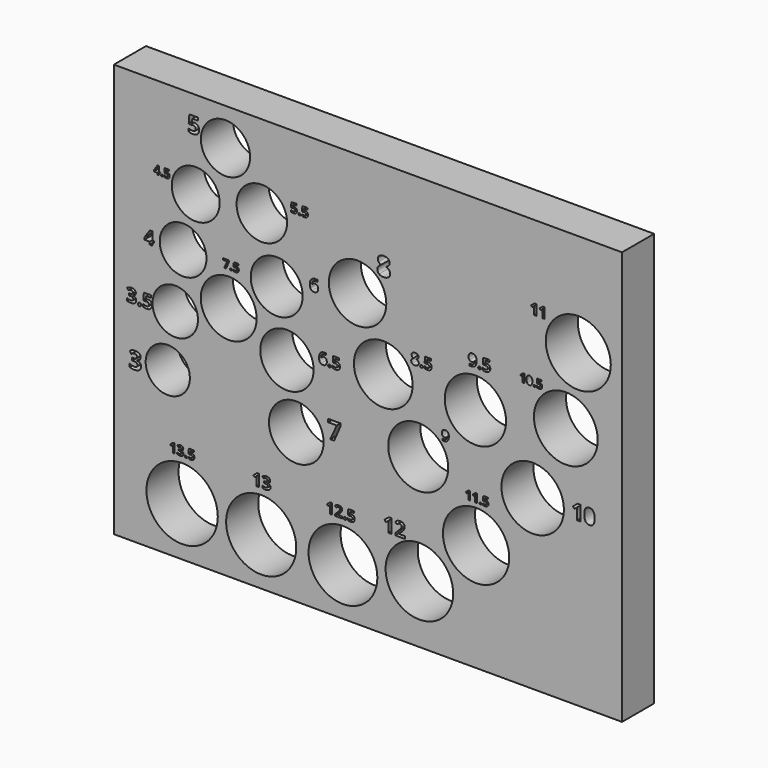
from build123d import *

# Parameters (mm, degrees)
F0_W     = 160.9384715557
F0_H     = 130.9329941869
F0_R     = 11.3
F0_R_2   = 11.1
F0_R_3   = 10.9
F0_R_4   = 7
F0_R_5   = 8.65
F0_R_6   = 10.7
F0_R_7   = 10.5
F0_R_8   = 9.5
F0_R_9   = 9.9
F0_R_10  = 7.2
F0_R_11  = 8.85
F0_R_12  = 7.4
F0_R_13  = 8.45
F0_R_14  = 8.225
F0_R_15  = 9.1
F0_R_16  = 7.6
F0_R_17  = 7.8
F0_R_18  = 8
F0_R_19  = 9.3
F0_R_20  = 9.7
F0_R_21  = 10.1
F0_R_22  = 10.3
F1_DEPTH = 12.7


with BuildPart() as f1:
    # F0 (on Front) → F1 (new body)
    with BuildSketch(Plane.XZ):
        with Locations((-0.597499311, -12.6713551581)):
            Rectangle(F0_W, F0_H)
        with Locations((-59.4613514841, -62.5652894378)):
            Circle(F0_R, mode=Mode.SUBTRACT)
        with BuildLine():
            Line((-61.8060982217, -46.5335902021), (-61.8060982217, -49.4282282889))
            Line((-61.8060982217, -49.4282282889), (-62.4180965565, -49.4282282889))
            Line((-62.4180965565, -49.4282282889), (-62.4180965565, -47.7531521012))
            Line((-62.4180965565, -47.7531521012), (-62.41176117, -47.4781963276))
            Line((-62.41176117, -47.4781963276), (-62.4022580903, -47.1772654693))
            add(Edge.make_bspline(
                [(-62.4022580903, -47.1772654693), (-62.554307366, -47.3293147451), (-62.613859999, -47.3768301438)],
                knots=[0, 0, 0, 1, 1, 1], degree=2))
            Line((-62.613859999, -47.3768301438), (-62.9464677897, -47.6441834536))
            Line((-62.9464677897, -47.6441834536), (-63.2416968001, -47.2760974986))
            Line((-63.2416968001, -47.2760974986), (-62.3091279089, -46.5335902021))
            Line((-62.3091279089, -46.5335902021), (-61.8060982217, -46.5335902021))
        make_face(mode=Mode.SUBTRACT)
        with BuildLine():
            add(Edge.make_bspline(
                [(-59.3543036505, -46.6745525514), (-59.0939192658, -46.856694913), (-59.0939192658, -47.1810667012)],
                knots=[0, 0, 0, 1, 1, 1], degree=2))
            add(Edge.make_bspline(
                [(-59.0939192658, -47.1810667012), (-59.0939192658, -47.452221243), (-59.2583225451, -47.6422828376)],
                knots=[0, 0, 0, 1, 1, 1], degree=2))
            add(Edge.make_bspline(
                [(-59.2583225451, -47.6422828376), (-59.4227258245, -47.8323444323), (-59.7198554509, -47.9039342996)],
                knots=[0, 0, 0, 1, 1, 1], degree=2))
            Line((-59.7198554509, -47.9039342996), (-59.7198554509, -47.9153379953))
            add(Edge.make_bspline(
                [(-59.7198554509, -47.9153379953), (-59.3688750394, -47.9590521621), (-59.1889500631, -48.1285237507)],
                knots=[0, 0, 0, 1, 1, 1], degree=2))
            add(Edge.make_bspline(
                [(-59.1889500631, -48.1285237507), (-59.0090250868, -48.2979953393), (-59.0090250868, -48.5849883472)],
                knots=[0, 0, 0, 1, 1, 1], degree=2))
            add(Edge.make_bspline(
                [(-59.0090250868, -48.5849883472), (-59.0090250868, -49.0024903168), (-59.311856561, -49.2353157703)],
                knots=[0, 0, 0, 1, 1, 1], degree=2))
            add(Edge.make_bspline(
                [(-59.311856561, -49.2353157703), (-59.6146880352, -49.4681412238), (-60.1766368167, -49.4681412238)],
                knots=[0, 0, 0, 1, 1, 1], degree=2))
            add(Edge.make_bspline(
                [(-60.1766368167, -49.4681412238), (-60.6479895715, -49.4681412238), (-61.0122742946, -49.3116571775)],
                knots=[0, 0, 0, 1, 1, 1], degree=2))
            Line((-61.0122742946, -49.3116571775), (-61.0122742946, -48.7908884081))
            add(Edge.make_bspline(
                [(-61.0122742946, -48.7908884081), (-60.8443865527, -48.875782587), (-60.6422877237, -48.9293166029)],
                knots=[0, 0, 0, 1, 1, 1], degree=2))
            add(Edge.make_bspline(
                [(-60.6422877237, -48.9293166029), (-60.4401888947, -48.9828506187), (-60.2425248362, -48.9828506187)],
                knots=[0, 0, 0, 1, 1, 1], degree=2))
            add(Edge.make_bspline(
                [(-60.2425248362, -48.9828506187), (-59.9390598234, -48.9828506187), (-59.7946130114, -48.8799005883)],
                knots=[0, 0, 0, 1, 1, 1], degree=2))
            add(Edge.make_bspline(
                [(-59.7946130114, -48.8799005883), (-59.6501661995, -48.7769505578), (-59.6501661995, -48.5488766442)],
                knots=[0, 0, 0, 1, 1, 1], degree=2))
            add(Edge.make_bspline(
                [(-59.6501661995, -48.5488766442), (-59.6501661995, -48.3455107379), (-59.8164700948, -48.2602997896)],
                knots=[0, 0, 0, 1, 1, 1], degree=2))
            add(Edge.make_bspline(
                [(-59.8164700948, -48.2602997896), (-59.9827739902, -48.1750888414), (-60.3470587133, -48.1750888414)],
                knots=[0, 0, 0, 1, 1, 1], degree=2))
            Line((-60.3470587133, -48.1750888414), (-60.5668966244, -48.1750888414))
            Line((-60.5668966244, -48.1750888414), (-60.5668966244, -47.7056367025))
            Line((-60.5668966244, -47.7056367025), (-60.3432574814, -47.7056367025))
            add(Edge.make_bspline(
                [(-60.3432574814, -47.7056367025), (-60.0068484588, -47.7056367025), (-59.8513147205, -47.6175748303)],
                knots=[0, 0, 0, 1, 1, 1], degree=2))
            add(Edge.make_bspline(
                [(-59.8513147205, -47.6175748303), (-59.6957809822, -47.5295129581), (-59.6957809822, -47.3160104335)],
                knots=[0, 0, 0, 1, 1, 1], degree=2))
            add(Edge.make_bspline(
                [(-59.6957809822, -47.3160104335), (-59.6957809822, -46.9872038747), (-60.107581104, -46.9872038747)],
                knots=[0, 0, 0, 1, 1, 1], degree=2))
            add(Edge.make_bspline(
                [(-60.107581104, -46.9872038747), (-60.2501273, -46.9872038747), (-60.3977418052, -47.0347192733)],
                knots=[0, 0, 0, 1, 1, 1], degree=2))
            add(Edge.make_bspline(
                [(-60.3977418052, -47.0347192733), (-60.5453563104, -47.082234672), (-60.7252812867, -47.1988057834)],
                knots=[0, 0, 0, 1, 1, 1], degree=2))
            Line((-60.7252812867, -47.1988057834), (-61.0084730627, -46.7775025819))
            add(Edge.make_bspline(
                [(-61.0084730627, -46.7775025819), (-60.6125114072, -46.4924101899), (-60.0638669372, -46.4924101899)],
                knots=[0, 0, 0, 1, 1, 1], degree=2))
            add(Edge.make_bspline(
                [(-60.0638669372, -46.4924101899), (-59.6146880352, -46.4924101899), (-59.3543036505, -46.6745525514)],
                knots=[0, 0, 0, 1, 1, 1], degree=2))
        make_face(mode=Mode.SUBTRACT)
        with BuildLine():
            add(Edge.make_bspline(
                [(-58.5297530989, -49.3933836632), (-58.620665895, -49.305321791), (-58.620665895, -49.1450365128)],
                knots=[0, 0, 0, 1, 1, 1], degree=2))
            add(Edge.make_bspline(
                [(-58.620665895, -49.1450365128), (-58.620665895, -48.9790493868), (-58.5316537149, -48.8938384385)],
                knots=[0, 0, 0, 1, 1, 1], degree=2))
            add(Edge.make_bspline(
                [(-58.5316537149, -48.8938384385), (-58.4426415347, -48.8086274903), (-58.2722196381, -48.8086274903)],
                knots=[0, 0, 0, 1, 1, 1], degree=2))
            add(Edge.make_bspline(
                [(-58.2722196381, -48.8086274903), (-58.1081331281, -48.8086274903), (-58.0181706399, -48.8957390545)],
                knots=[0, 0, 0, 1, 1, 1], degree=2))
            add(Edge.make_bspline(
                [(-58.0181706399, -48.8957390545), (-57.9282081518, -48.9828506187), (-57.9282081518, -49.1450365128)],
                knots=[0, 0, 0, 1, 1, 1], degree=2))
            add(Edge.make_bspline(
                [(-57.9282081518, -49.1450365128), (-57.9282081518, -49.3015205591), (-58.0191209479, -49.3914830473)],
                knots=[0, 0, 0, 1, 1, 1], degree=2))
            add(Edge.make_bspline(
                [(-58.0191209479, -49.3914830473), (-58.110033744, -49.4814455354), (-58.2722196381, -49.4814455354)],
                knots=[0, 0, 0, 1, 1, 1], degree=2))
            add(Edge.make_bspline(
                [(-58.2722196381, -49.4814455354), (-58.4388403028, -49.4814455354), (-58.5297530989, -49.3933836632)],
                knots=[0, 0, 0, 1, 1, 1], degree=2))
        make_face(mode=Mode.SUBTRACT)
        with BuildLine():
            add(Edge.make_bspline(
                [(-56.7796025813, -47.6068046733), (-56.6585966994, -47.5789289727), (-56.480572339, -47.5789289727)],
                knots=[0, 0, 0, 1, 1, 1], degree=2))
            add(Edge.make_bspline(
                [(-56.480572339, -47.5789289727), (-56.0611697535, -47.5789289727), (-55.8125058338, -47.8146053501)],
                knots=[0, 0, 0, 1, 1, 1], degree=2))
            add(Edge.make_bspline(
                [(-55.8125058338, -47.8146053501), (-55.5638419141, -48.0502817275), (-55.5638419141, -48.4601812334)],
                knots=[0, 0, 0, 1, 1, 1], degree=2))
            add(Edge.make_bspline(
                [(-55.5638419141, -48.4601812334), (-55.5638419141, -48.9448382998), (-55.8628721564, -49.2064897618)],
                knots=[0, 0, 0, 1, 1, 1], degree=2))
            add(Edge.make_bspline(
                [(-55.8628721564, -49.2064897618), (-56.1619023986, -49.4681412238), (-56.7181493324, -49.4681412238)],
                knots=[0, 0, 0, 1, 1, 1], degree=2))
            add(Edge.make_bspline(
                [(-56.7181493324, -49.4681412238), (-57.2015393215, -49.4681412238), (-57.4980354092, -49.3116571775)],
                knots=[0, 0, 0, 1, 1, 1], degree=2))
            Line((-57.4980354092, -49.3116571775), (-57.4980354092, -48.7826524057))
            add(Edge.make_bspline(
                [(-57.4980354092, -48.7826524057), (-57.3421849015, -48.8656459687), (-57.1340674554, -48.9182296765)],
                knots=[0, 0, 0, 1, 1, 1], degree=2))
            add(Edge.make_bspline(
                [(-57.1340674554, -48.9182296765), (-56.9259500092, -48.9708133844), (-56.7403231851, -48.9708133844)],
                knots=[0, 0, 0, 1, 1, 1], degree=2))
            add(Edge.make_bspline(
                [(-56.7403231851, -48.9708133844), (-56.1796414808, -48.9708133844), (-56.1796414808, -48.5114978639)],
                knots=[0, 0, 0, 1, 1, 1], degree=2))
            add(Edge.make_bspline(
                [(-56.1796414808, -48.5114978639), (-56.1796414808, -48.0737226575), (-56.7599628832, -48.0737226575)],
                knots=[0, 0, 0, 1, 1, 1], degree=2))
            add(Edge.make_bspline(
                [(-56.7599628832, -48.0737226575), (-56.8644967603, -48.0737226575), (-56.9912044901, -48.094629433)],
                knots=[0, 0, 0, 1, 1, 1], degree=2))
            add(Edge.make_bspline(
                [(-56.9912044901, -48.094629433), (-57.1179122198, -48.1155362084), (-57.1971045509, -48.139610677)],
                knots=[0, 0, 0, 1, 1, 1], degree=2))
            Line((-57.1971045509, -48.139610677), (-57.4410169308, -48.0084681767))
            Line((-57.4410169308, -48.0084681767), (-57.3320482832, -46.5335902021))
            Line((-57.3320482832, -46.5335902021), (-55.7621395112, -46.5335902021))
            Line((-55.7621395112, -46.5335902021), (-55.7621395112, -47.0524583555))
            Line((-55.7621395112, -47.0524583555), (-56.7954410475, -47.0524583555))
            Line((-56.7954410475, -47.0524583555), (-56.8486582941, -47.6207425236))
            Line((-56.8486582941, -47.6207425236), (-56.7796025813, -47.6068046733))
        make_face(mode=Mode.SUBTRACT)
        with Locations((-34.4101041555, -63.1219893694)):
            Circle(F0_R_2, mode=Mode.SUBTRACT)
        with Locations((-8.5238143802, -63.1219893694)):
            Circle(F0_R_3, mode=Mode.SUBTRACT)
        with BuildLine():
            Line((-35.0533799792, -46.3321228235), (-35.0533799792, -50.0538051128))
            Line((-35.0533799792, -50.0538051128), (-35.8402359852, -50.0538051128))
            Line((-35.8402359852, -50.0538051128), (-35.8402359852, -47.9001329804))
            Line((-35.8402359852, -47.9001329804), (-35.8320904779, -47.5466179632))
            Line((-35.8320904779, -47.5466179632), (-35.819872217, -47.1597063661))
            add(Edge.make_bspline(
                [(-35.819872217, -47.1597063661), (-36.0153643924, -47.3551985415), (-36.0919321611, -47.4162898463)],
                knots=[0, 0, 0, 1, 1, 1], degree=2))
            Line((-36.0919321611, -47.4162898463), (-36.5195712948, -47.7600302547))
            Line((-36.5195712948, -47.7600302547), (-36.8991519354, -47.2867762801))
            Line((-36.8991519354, -47.2867762801), (-35.7001332595, -46.3321228235))
            Line((-35.7001332595, -46.3321228235), (-35.0533799792, -46.3321228235))
        make_face(mode=Mode.SUBTRACT)
        with BuildLine():
            add(Edge.make_bspline(
                [(-31.9010686508, -46.5133603611), (-31.5662883004, -46.7475436963), (-31.5662883004, -47.1645936705)],
                knots=[0, 0, 0, 1, 1, 1], degree=2))
            add(Edge.make_bspline(
                [(-31.5662883004, -47.1645936705), (-31.5662883004, -47.5132213833), (-31.777664215, -47.7575866025)],
                knots=[0, 0, 0, 1, 1, 1], degree=2))
            add(Edge.make_bspline(
                [(-31.777664215, -47.7575866025), (-31.9890401297, -48.0019518218), (-32.3710644225, -48.0939960544)],
                knots=[0, 0, 0, 1, 1, 1], degree=2))
            Line((-32.3710644225, -48.0939960544), (-32.3710644225, -48.1086579675))
            add(Edge.make_bspline(
                [(-32.3710644225, -48.1086579675), (-31.9198033176, -48.164861968), (-31.68847091, -48.3827542885)],
                knots=[0, 0, 0, 1, 1, 1], degree=2))
            add(Edge.make_bspline(
                [(-31.68847091, -48.3827542885), (-31.4571385024, -48.600646609), (-31.4571385024, -48.9696380901)],
                knots=[0, 0, 0, 1, 1, 1], degree=2))
            add(Edge.make_bspline(
                [(-31.4571385024, -48.9696380901), (-31.4571385024, -49.5064270217), (-31.8464937518, -49.8057744153)],
                knots=[0, 0, 0, 1, 1, 1], degree=2))
            add(Edge.make_bspline(
                [(-31.8464937518, -49.8057744153), (-32.2358490012, -50.1051218089), (-32.9583554994, -50.1051218089)],
                knots=[0, 0, 0, 1, 1, 1], degree=2))
            add(Edge.make_bspline(
                [(-32.9583554994, -50.1051218089), (-33.5643812432, -50.1051218089), (-34.0327479134, -49.9039277784)],
                knots=[0, 0, 0, 1, 1, 1], degree=2))
            Line((-34.0327479134, -49.9039277784), (-34.0327479134, -49.2343670776))
            add(Edge.make_bspline(
                [(-34.0327479134, -49.2343670776), (-33.8168919698, -49.3435168755), (-33.5570502866, -49.4123464123)],
                knots=[0, 0, 0, 1, 1, 1], degree=2))
            add(Edge.make_bspline(
                [(-33.5570502866, -49.4123464123), (-33.2972086035, -49.481175949), (-33.0430687754, -49.481175949)],
                knots=[0, 0, 0, 1, 1, 1], degree=2))
            add(Edge.make_bspline(
                [(-33.0430687754, -49.481175949), (-32.6528989754, -49.481175949), (-32.4671814087, -49.3488114553)],
                knots=[0, 0, 0, 1, 1, 1], degree=2))
            add(Edge.make_bspline(
                [(-32.4671814087, -49.3488114553), (-32.2814638421, -49.2164469615), (-32.2814638421, -48.9232086984)],
                knots=[0, 0, 0, 1, 1, 1], degree=2))
            add(Edge.make_bspline(
                [(-32.2814638421, -48.9232086984), (-32.2814638421, -48.6617379138), (-32.4952834089, -48.5521808405)],
                knots=[0, 0, 0, 1, 1, 1], degree=2))
            add(Edge.make_bspline(
                [(-32.4952834089, -48.5521808405), (-32.7091029758, -48.4426237672), (-33.177469646, -48.4426237672)],
                knots=[0, 0, 0, 1, 1, 1], degree=2))
            Line((-33.177469646, -48.4426237672), (-33.4601187496, -48.4426237672))
            Line((-33.4601187496, -48.4426237672), (-33.4601187496, -47.8390416756))
            Line((-33.4601187496, -47.8390416756), (-33.1725823416, -47.8390416756))
            add(Edge.make_bspline(
                [(-33.1725823416, -47.8390416756), (-32.7400559036, -47.8390416756), (-32.5400836991, -47.725819124)],
                knots=[0, 0, 0, 1, 1, 1], degree=2))
            add(Edge.make_bspline(
                [(-32.5400836991, -47.725819124), (-32.3401114947, -47.6125965724), (-32.3401114947, -47.3380929761)],
                knots=[0, 0, 0, 1, 1, 1], degree=2))
            add(Edge.make_bspline(
                [(-32.3401114947, -47.3380929761), (-32.3401114947, -46.9153411468), (-32.8695694698, -46.9153411468)],
                knots=[0, 0, 0, 1, 1, 1], degree=2))
            add(Edge.make_bspline(
                [(-32.8695694698, -46.9153411468), (-33.0528433842, -46.9153411468), (-33.2426337045, -46.9764324516)],
                knots=[0, 0, 0, 1, 1, 1], degree=2))
            add(Edge.make_bspline(
                [(-33.2426337045, -46.9764324516), (-33.4324240248, -47.0375237564), (-33.6637564324, -47.1874010909)],
                knots=[0, 0, 0, 1, 1, 1], degree=2))
            Line((-33.6637564324, -47.1874010909), (-34.0278606091, -46.6457248549))
            add(Edge.make_bspline(
                [(-34.0278606091, -46.6457248549), (-33.5187664023, -46.279177026), (-32.8133654693, -46.279177026)],
                knots=[0, 0, 0, 1, 1, 1], degree=2))
            add(Edge.make_bspline(
                [(-32.8133654693, -46.279177026), (-32.2358490012, -46.279177026), (-31.9010686508, -46.5133603611)],
                knots=[0, 0, 0, 1, 1, 1], degree=2))
        make_face(mode=Mode.SUBTRACT)
        with BuildLine():
            Line((-11.9379018854, -46.9541698961), (-11.9379018854, -50.2623282373))
            Line((-11.9379018854, -50.2623282373), (-12.6373286653, -50.2623282373))
            Line((-12.6373286653, -50.2623282373), (-12.6373286653, -48.347955146))
            Line((-12.6373286653, -48.347955146), (-12.6300882225, -48.033719926))
            Line((-12.6300882225, -48.033719926), (-12.6192275582, -47.6897988903))
            add(Edge.make_bspline(
                [(-12.6192275582, -47.6897988903), (-12.7929981867, -47.8635695189), (-12.8610583496, -47.9178728403)],
                knots=[0, 0, 0, 1, 1, 1], degree=2))
            Line((-12.8610583496, -47.9178728403), (-13.2411815996, -48.2234195289))
            Line((-13.2411815996, -48.2234195289), (-13.5785862367, -47.8027497989))
            Line((-13.5785862367, -47.8027497989), (-12.5127930482, -46.9541698961))
            Line((-12.5127930482, -46.9541698961), (-11.9379018854, -46.9541698961))
        make_face(mode=Mode.SUBTRACT)
        with BuildLine():
            add(Edge.make_bspline(
                [(-8.1935068621, -50.2225058016), (-8.2974072171, -50.1218636459), (-8.2974072171, -49.9386804416)],
                knots=[0, 0, 0, 1, 1, 1], degree=2))
            add(Edge.make_bspline(
                [(-8.2974072171, -49.9386804416), (-8.2974072171, -49.7489808388), (-8.1956789949, -49.6515968823)],
                knots=[0, 0, 0, 1, 1, 1], degree=2))
            add(Edge.make_bspline(
                [(-8.1956789949, -49.6515968823), (-8.0939507728, -49.5542129259), (-7.89918286, -49.5542129259)],
                knots=[0, 0, 0, 1, 1, 1], degree=2))
            add(Edge.make_bspline(
                [(-7.89918286, -49.5542129259), (-7.71165539, -49.5542129259), (-7.6088411014, -49.6537690152)],
                knots=[0, 0, 0, 1, 1, 1], degree=2))
            add(Edge.make_bspline(
                [(-7.6088411014, -49.6537690152), (-7.5060268128, -49.7533251045), (-7.5060268128, -49.9386804416)],
                knots=[0, 0, 0, 1, 1, 1], degree=2))
            add(Edge.make_bspline(
                [(-7.5060268128, -49.9386804416), (-7.5060268128, -50.1175193802), (-7.6099271678, -50.2203336687)],
                knots=[0, 0, 0, 1, 1, 1], degree=2))
            add(Edge.make_bspline(
                [(-7.6099271678, -50.2203336687), (-7.7138275228, -50.3231479573), (-7.89918286, -50.3231479573)],
                knots=[0, 0, 0, 1, 1, 1], degree=2))
            add(Edge.make_bspline(
                [(-7.89918286, -50.3231479573), (-8.0896065071, -50.3231479573), (-8.1935068621, -50.2225058016)],
                knots=[0, 0, 0, 1, 1, 1], degree=2))
        make_face(mode=Mode.SUBTRACT)
        with BuildLine():
            Line((-8.7093884156, -49.6736802331), (-8.7093884156, -50.2623282373))
            Line((-8.7093884156, -50.2623282373), (-11.021985864, -50.2623282373))
            Line((-11.021985864, -50.2623282373), (-11.021985864, -49.7757704773))
            Line((-11.021985864, -49.7757704773), (-10.1915070684, -48.9366031502))
            add(Edge.make_bspline(
                [(-10.1915070684, -48.9366031502), (-9.8222444827, -48.5586520331), (-9.7092935741, -48.4127571096)],
                knots=[0, 0, 0, 1, 1, 1], degree=2))
            add(Edge.make_bspline(
                [(-9.7092935741, -48.4127571096), (-9.5963426655, -48.266862186), (-9.5463836098, -48.1423265689)],
                knots=[0, 0, 0, 1, 1, 1], degree=2))
            add(Edge.make_bspline(
                [(-9.5463836098, -48.1423265689), (-9.4964245541, -48.0177909517), (-9.4964245541, -47.8845668032)],
                knots=[0, 0, 0, 1, 1, 1], degree=2))
            add(Edge.make_bspline(
                [(-9.4964245541, -47.8845668032), (-9.4964245541, -47.6854546246), (-9.6064792855, -47.5880706682)],
                knots=[0, 0, 0, 1, 1, 1], degree=2))
            add(Edge.make_bspline(
                [(-9.6064792855, -47.5880706682), (-9.716534017, -47.4906867118), (-9.8997172212, -47.4906867118)],
                knots=[0, 0, 0, 1, 1, 1], degree=2))
            add(Edge.make_bspline(
                [(-9.8997172212, -47.4906867118), (-10.0915889569, -47.4906867118), (-10.2726000284, -47.5790201146)],
                knots=[0, 0, 0, 1, 1, 1], degree=2))
            add(Edge.make_bspline(
                [(-10.2726000284, -47.5790201146), (-10.4536110998, -47.6673535175), (-10.6505511455, -47.8302634818)],
                knots=[0, 0, 0, 1, 1, 1], degree=2))
            Line((-10.6505511455, -47.8302634818), (-11.0306743954, -47.3799079361))
            add(Edge.make_bspline(
                [(-11.0306743954, -47.3799079361), (-10.7866714712, -47.1713831818), (-10.6259336398, -47.0855839339)],
                knots=[0, 0, 0, 1, 1, 1], degree=2))
            add(Edge.make_bspline(
                [(-10.6259336398, -47.0855839339), (-10.4651958083, -46.9997846861), (-10.2751341834, -46.9534458518)],
                knots=[0, 0, 0, 1, 1, 1], degree=2))
            add(Edge.make_bspline(
                [(-10.2751341834, -46.9534458518), (-10.0850725584, -46.9071070175), (-9.8497581655, -46.9071070175)],
                knots=[0, 0, 0, 1, 1, 1], degree=2))
            add(Edge.make_bspline(
                [(-9.8497581655, -46.9071070175), (-9.5398672113, -46.9071070175), (-9.3023806856, -47.0200579261)],
                knots=[0, 0, 0, 1, 1, 1], degree=2))
            add(Edge.make_bspline(
                [(-9.3023806856, -47.0200579261), (-9.0648941599, -47.1330088347), (-8.933480122, -47.3368273011)],
                knots=[0, 0, 0, 1, 1, 1], degree=2))
            add(Edge.make_bspline(
                [(-8.933480122, -47.3368273011), (-8.8020660842, -47.5406457675), (-8.8020660842, -47.8027497989)],
                knots=[0, 0, 0, 1, 1, 1], degree=2))
            add(Edge.make_bspline(
                [(-8.8020660842, -47.8027497989), (-8.8020660842, -48.0315477932), (-8.8824349999, -48.2317460382)],
                knots=[0, 0, 0, 1, 1, 1], degree=2))
            add(Edge.make_bspline(
                [(-8.8824349999, -48.2317460382), (-8.9628039156, -48.4319442831), (-9.1315062341, -48.6422791481)],
                knots=[0, 0, 0, 1, 1, 1], degree=2))
            add(Edge.make_bspline(
                [(-9.1315062341, -48.6422791481), (-9.3002085527, -48.8526140131), (-9.7252225484, -49.2421498388)],
                knots=[0, 0, 0, 1, 1, 1], degree=2))
            Line((-9.7252225484, -49.2421498388), (-10.1509605884, -49.6425463288))
            Line((-10.1509605884, -49.6425463288), (-10.1509605884, -49.6736802331))
            Line((-10.1509605884, -49.6736802331), (-8.7093884156, -49.6736802331))
        make_face(mode=Mode.SUBTRACT)
        with BuildLine():
            add(Edge.make_bspline(
                [(-6.1933345229, -48.180700916), (-6.0550420644, -48.1488429674), (-5.8515856201, -48.1488429674)],
                knots=[0, 0, 0, 1, 1, 1], degree=2))
            add(Edge.make_bspline(
                [(-5.8515856201, -48.1488429674), (-5.372268303, -48.1488429674), (-5.0880809209, -48.4181874417)],
                knots=[0, 0, 0, 1, 1, 1], degree=2))
            add(Edge.make_bspline(
                [(-5.0880809209, -48.4181874417), (-4.8038935387, -48.687531916), (-4.8038935387, -49.1559885688)],
                knots=[0, 0, 0, 1, 1, 1], degree=2))
            add(Edge.make_bspline(
                [(-4.8038935387, -49.1559885688), (-4.8038935387, -49.7098824473), (-5.1456424416, -50.0089127373)],
                knots=[0, 0, 0, 1, 1, 1], degree=2))
            add(Edge.make_bspline(
                [(-5.1456424416, -50.0089127373), (-5.4873913444, -50.3079430273), (-6.1231022272, -50.3079430273)],
                knots=[0, 0, 0, 1, 1, 1], degree=2))
            add(Edge.make_bspline(
                [(-6.1231022272, -50.3079430273), (-6.6755480172, -50.3079430273), (-7.0144007429, -50.1291040887)],
                knots=[0, 0, 0, 1, 1, 1], degree=2))
            Line((-7.0144007429, -50.1291040887), (-7.0144007429, -49.5245271102))
            add(Edge.make_bspline(
                [(-7.0144007429, -49.5245271102), (-6.8362858486, -49.6193769116), (-6.5984373008, -49.6794725873)],
                knots=[0, 0, 0, 1, 1, 1], degree=2))
            add(Edge.make_bspline(
                [(-6.5984373008, -49.6794725873), (-6.3605887529, -49.739568263), (-6.1484437772, -49.739568263)],
                knots=[0, 0, 0, 1, 1, 1], degree=2))
            add(Edge.make_bspline(
                [(-6.1484437772, -49.739568263), (-5.5076645844, -49.739568263), (-5.5076645844, -49.2146361559)],
                knots=[0, 0, 0, 1, 1, 1], degree=2))
            add(Edge.make_bspline(
                [(-5.5076645844, -49.2146361559), (-5.5076645844, -48.7143215545), (-6.1708891501, -48.7143215545)],
                knots=[0, 0, 0, 1, 1, 1], degree=2))
            add(Edge.make_bspline(
                [(-6.1708891501, -48.7143215545), (-6.2903564572, -48.7143215545), (-6.4351653143, -48.738215016)],
                knots=[0, 0, 0, 1, 1, 1], degree=2))
            add(Edge.make_bspline(
                [(-6.4351653143, -48.738215016), (-6.5799741715, -48.7621084774), (-6.6704797072, -48.7896221603)],
                knots=[0, 0, 0, 1, 1, 1], degree=2))
            Line((-6.6704797072, -48.7896221603), (-6.9492367572, -48.6397449931))
            Line((-6.9492367572, -48.6397449931), (-6.82470114, -46.9541698961))
            Line((-6.82470114, -46.9541698961), (-5.0305194002, -46.9541698961))
            Line((-5.0305194002, -46.9541698961), (-5.0305194002, -47.5471621661))
            Line((-5.0305194002, -47.5471621661), (-6.2114356301, -47.5471621661))
            Line((-6.2114356301, -47.5471621661), (-6.2722553501, -48.1966298903))
            Line((-6.2722553501, -48.1966298903), (-6.1933345229, -48.180700916))
        make_face(mode=Mode.SUBTRACT)
        with BuildLine():
            add(Edge.make_bspline(
                [(-73.0627112247, -25.13195103), (-72.5910069175, -25.4619145053), (-72.5910069175, -26.049536416)],
                knots=[0, 0, 0, 1, 1, 1], degree=2))
            add(Edge.make_bspline(
                [(-72.5910069175, -26.049536416), (-72.5910069175, -26.540751607), (-72.8888348195, -26.8850613203)],
                knots=[0, 0, 0, 1, 1, 1], degree=2))
            add(Edge.make_bspline(
                [(-72.8888348195, -26.8850613203), (-73.1866627215, -27.2293710336), (-73.7249335733, -27.3590610256)],
                knots=[0, 0, 0, 1, 1, 1], degree=2))
            Line((-73.7249335733, -27.3590610256), (-73.7249335733, -27.3797196084))
            add(Edge.make_bspline(
                [(-73.7249335733, -27.3797196084), (-73.0891083028, -27.4589108424), (-72.7631617742, -27.7659203368)],
                knots=[0, 0, 0, 1, 1, 1], degree=2))
            add(Edge.make_bspline(
                [(-72.7631617742, -27.7659203368), (-72.4372152456, -28.0729298312), (-72.4372152456, -28.5928374983)],
                knots=[0, 0, 0, 1, 1, 1], degree=2))
            add(Edge.make_bspline(
                [(-72.4372152456, -28.5928374983), (-72.4372152456, -29.3491711685), (-72.9858153888, -29.7709505673)],
                knots=[0, 0, 0, 1, 1, 1], degree=2))
            add(Edge.make_bspline(
                [(-72.9858153888, -29.7709505673), (-73.534415532, -30.1927299661), (-74.5524245843, -30.1927299661)],
                knots=[0, 0, 0, 1, 1, 1], degree=2))
            add(Edge.make_bspline(
                [(-74.5524245843, -30.1927299661), (-75.4063126733, -30.1927299661), (-76.0662396238, -29.9092483021)],
                knots=[0, 0, 0, 1, 1, 1], degree=2))
            Line((-76.0662396238, -29.9092483021), (-76.0662396238, -28.9658396877))
            add(Edge.make_bspline(
                [(-76.0662396238, -28.9658396877), (-75.762099377, -29.1196313596), (-75.3959833819, -29.2166119289)],
                knots=[0, 0, 0, 1, 1, 1], degree=2))
            add(Edge.make_bspline(
                [(-75.3959833819, -29.2166119289), (-75.0298673867, -29.3135924981), (-74.6717852849, -29.3135924981)],
                knots=[0, 0, 0, 1, 1, 1], degree=2))
            add(Edge.make_bspline(
                [(-74.6717852849, -29.3135924981), (-74.1220374427, -29.3135924981), (-73.8603620606, -29.1270914034)],
                knots=[0, 0, 0, 1, 1, 1], degree=2))
            add(Edge.make_bspline(
                [(-73.8603620606, -29.1270914034), (-73.5986866785, -28.9405903087), (-73.5986866785, -28.5274186527)],
                knots=[0, 0, 0, 1, 1, 1], degree=2))
            add(Edge.make_bspline(
                [(-73.5986866785, -28.5274186527), (-73.5986866785, -28.1590072595), (-73.8999576776, -28.004641738)],
                knots=[0, 0, 0, 1, 1, 1], degree=2))
            add(Edge.make_bspline(
                [(-73.8999576776, -28.004641738), (-74.2012286767, -27.8502762166), (-74.8611556272, -27.8502762166)],
                knots=[0, 0, 0, 1, 1, 1], degree=2))
            Line((-74.8611556272, -27.8502762166), (-75.2594071956, -27.8502762166))
            Line((-75.2594071956, -27.8502762166), (-75.2594071956, -26.9998312247))
            Line((-75.2594071956, -26.9998312247), (-74.854269433, -26.9998312247))
            add(Edge.make_bspline(
                [(-74.854269433, -26.9998312247), (-74.2448412404, -26.9998312247), (-73.963081125, -26.8403010575)],
                knots=[0, 0, 0, 1, 1, 1], degree=2))
            add(Edge.make_bspline(
                [(-73.963081125, -26.8403010575), (-73.6813210096, -26.6807708904), (-73.6813210096, -26.2939963124)],
                knots=[0, 0, 0, 1, 1, 1], degree=2))
            add(Edge.make_bspline(
                [(-73.6813210096, -26.2939963124), (-73.6813210096, -25.6983405084), (-74.4273253885, -25.6983405084)],
                knots=[0, 0, 0, 1, 1, 1], degree=2))
            add(Edge.make_bspline(
                [(-74.4273253885, -25.6983405084), (-74.6855576734, -25.6983405084), (-74.9529715508, -25.7844179367)],
                knots=[0, 0, 0, 1, 1, 1], degree=2))
            add(Edge.make_bspline(
                [(-74.9529715508, -25.7844179367), (-75.2203854281, -25.8704953651), (-75.5463319567, -26.0816719892)],
                knots=[0, 0, 0, 1, 1, 1], degree=2))
            Line((-75.5463319567, -26.0816719892), (-76.0593534295, -25.3184521247))
            add(Edge.make_bspline(
                [(-76.0593534295, -25.3184521247), (-75.3420415268, -24.8019875548), (-74.3481341544, -24.8019875548)],
                knots=[0, 0, 0, 1, 1, 1], degree=2))
            add(Edge.make_bspline(
                [(-74.3481341544, -24.8019875548), (-73.534415532, -24.8019875548), (-73.0627112247, -25.13195103)],
                knots=[0, 0, 0, 1, 1, 1], degree=2))
        make_face(mode=Mode.SUBTRACT)
        with Locations((-63.9995783567, -26.8082283437)):
            Circle(F0_R_4, mode=Mode.SUBTRACT)
        with Locations((-23.3035776764, -30.936807394)):
            Circle(F0_R_5, mode=Mode.SUBTRACT)
        Polygon((-11.3210844841, -29.3962862343), (-12.5448942906, -29.3962862343), (-10.4717870567, -24.8658945517), (-13.1936463796, -24.8658945517), (-13.1936463796, -23.8837056349), (-9.2334799968, -23.8837056349), (-9.2334799968, -24.6170250353), align=None, mode=Mode.SUBTRACT)
        with Locations((15.6923905015, -59.781819582)):
            Circle(F0_R_6, mode=Mode.SUBTRACT)
        with BuildLine():
            Line((6.8355402683, -45.0671095581), (6.8355402683, -49.4829751551))
            Line((6.8355402683, -49.4829751551), (5.9019166818, -49.4829751551))
            Line((5.9019166818, -49.4829751551), (5.9019166818, -46.9275913428))
            Line((5.9019166818, -46.9275913428), (5.9115815222, -46.5081372677))
            Line((5.9115815222, -46.5081372677), (5.9260787829, -46.0490573468))
            add(Edge.make_bspline(
                [(5.9260787829, -46.0490573468), (5.6941226123, -46.2810135173), (5.6032731122, -46.3534998206)],
                knots=[0, 0, 0, 1, 1, 1], degree=2))
            Line((5.6032731122, -46.3534998206), (5.0958689891, -46.7613560872))
            Line((5.0958689891, -46.7613560872), (4.6454874246, -46.1998288576))
            Line((4.6454874246, -46.1998288576), (6.0681519373, -45.0671095581))
            Line((6.0681519373, -45.0671095581), (6.8355402683, -45.0671095581))
        make_face(mode=Mode.SUBTRACT)
        with BuildLine():
            Line((11.1450926205, -48.6972236273), (11.1450926205, -49.4829751551))
            Line((11.1450926205, -49.4829751551), (8.058142584, -49.4829751551))
            Line((8.058142584, -49.4829751551), (8.058142584, -48.8334978775))
            Line((8.058142584, -48.8334978775), (9.1666997824, -47.7133428705))
            add(Edge.make_bspline(
                [(9.1666997824, -47.7133428705), (9.6596066449, -47.2088381996), (9.8103781557, -47.0140916647)],
                knots=[0, 0, 0, 1, 1, 1], degree=2))
            add(Edge.make_bspline(
                [(9.8103781557, -47.0140916647), (9.9611496666, -46.8193451298), (10.0278370656, -46.6531098743)],
                knots=[0, 0, 0, 1, 1, 1], degree=2))
            add(Edge.make_bspline(
                [(10.0278370656, -46.6531098743), (10.0945244647, -46.4868746187), (10.0945244647, -46.3090415546)],
                knots=[0, 0, 0, 1, 1, 1], degree=2))
            add(Edge.make_bspline(
                [(10.0945244647, -46.3090415546), (10.0945244647, -46.0432584425), (9.94761889, -45.9132663386)],
                knots=[0, 0, 0, 1, 1, 1], degree=2))
            add(Edge.make_bspline(
                [(9.94761889, -45.9132663386), (9.8007133153, -45.7832742347), (9.5561928522, -45.7832742347)],
                knots=[0, 0, 0, 1, 1, 1], degree=2))
            add(Edge.make_bspline(
                [(9.5561928522, -45.7832742347), (9.3000745805, -45.7832742347), (9.0584535695, -45.901185288)],
                knots=[0, 0, 0, 1, 1, 1], degree=2))
            add(Edge.make_bspline(
                [(9.0584535695, -45.901185288), (8.8168325585, -46.0190963414), (8.5539488985, -46.2365552513)],
                knots=[0, 0, 0, 1, 1, 1], degree=2))
            Line((8.5539488985, -46.2365552513), (8.0465447754, -45.6354021759))
            add(Edge.make_bspline(
                [(8.0465447754, -45.6354021759), (8.3722498983, -45.3570547713), (8.586809356, -45.242526412)],
                knots=[0, 0, 0, 1, 1, 1], degree=2))
            add(Edge.make_bspline(
                [(8.586809356, -45.242526412), (8.8013688138, -45.1279980528), (9.0550708753, -45.066143074)],
                knots=[0, 0, 0, 1, 1, 1], degree=2))
            add(Edge.make_bspline(
                [(9.0550708753, -45.066143074), (9.3087729369, -45.0042880952), (9.6228802512, -45.0042880952)],
                knots=[0, 0, 0, 1, 1, 1], degree=2))
            add(Edge.make_bspline(
                [(9.6228802512, -45.0042880952), (10.036535422, -45.0042880952), (10.3535421885, -45.1550596061)],
                knots=[0, 0, 0, 1, 1, 1], degree=2))
            add(Edge.make_bspline(
                [(10.3535421885, -45.1550596061), (10.6705489549, -45.3058311169), (10.8459658089, -45.5778963753)],
                knots=[0, 0, 0, 1, 1, 1], degree=2))
            add(Edge.make_bspline(
                [(10.8459658089, -45.5778963753), (11.0213826629, -45.8499616337), (11.0213826629, -46.1998288576)],
                knots=[0, 0, 0, 1, 1, 1], degree=2))
            add(Edge.make_bspline(
                [(11.0213826629, -46.1998288576), (11.0213826629, -46.5052378155), (10.914102934, -46.7724706537)],
                knots=[0, 0, 0, 1, 1, 1], degree=2))
            add(Edge.make_bspline(
                [(10.914102934, -46.7724706537), (10.8068232051, -47.0397034919), (10.5816324229, -47.3204671067)],
                knots=[0, 0, 0, 1, 1, 1], degree=2))
            add(Edge.make_bspline(
                [(10.5816324229, -47.3204671067), (10.3564416406, -47.6012307214), (9.7891155068, -48.1211991371)],
                knots=[0, 0, 0, 1, 1, 1], degree=2))
            Line((9.7891155068, -48.1211991371), (9.2208228889, -48.6556648134))
            Line((9.2208228889, -48.6556648134), (9.2208228889, -48.6972236273))
            Line((9.2208228889, -48.6972236273), (11.1450926205, -48.6972236273))
        make_face(mode=Mode.SUBTRACT)
        with Locations((33.639062196, -43.9660288393)):
            Circle(F0_R_7, mode=Mode.SUBTRACT)
        with BuildLine():
            Line((31.7717184888, -29.3922340813), (31.7717184888, -32.0801138878))
            Line((31.7717184888, -32.0801138878), (31.2034339861, -32.0801138878))
            Line((31.2034339861, -32.0801138878), (31.2034339861, -30.5246850831))
            Line((31.2034339861, -30.5246850831), (31.2093168484, -30.2693688573))
            Line((31.2093168484, -30.2693688573), (31.2181411419, -29.9899328958))
            add(Edge.make_bspline(
                [(31.2181411419, -29.9899328958), (31.0769524456, -30.1311215921), (31.0216535395, -30.1752430597)],
                knots=[0, 0, 0, 1, 1, 1], degree=2))
            Line((31.0216535395, -30.1752430597), (30.7128032663, -30.4234998508))
            Line((30.7128032663, -30.4234998508), (30.4386618809, -30.0817055484))
            Line((30.4386618809, -30.0817055484), (31.3046192184, -29.3922340813))
            Line((31.3046192184, -29.3922340813), (31.7717184888, -29.3922340813))
        make_face(mode=Mode.SUBTRACT)
        with BuildLine():
            Line((33.9207281043, -29.3922340813), (33.9207281043, -32.0801138878))
            Line((33.9207281043, -32.0801138878), (33.3524436016, -32.0801138878))
            Line((33.3524436016, -32.0801138878), (33.3524436016, -30.5246850831))
            Line((33.3524436016, -30.5246850831), (33.3583264639, -30.2693688573))
            Line((33.3583264639, -30.2693688573), (33.3671507574, -29.9899328958))
            add(Edge.make_bspline(
                [(33.3671507574, -29.9899328958), (33.2259620611, -30.1311215921), (33.170663155, -30.1752430597)],
                knots=[0, 0, 0, 1, 1, 1], degree=2))
            Line((33.170663155, -30.1752430597), (32.8618128818, -30.4234998508))
            Line((32.8618128818, -30.4234998508), (32.5876714964, -30.0817055484))
            Line((32.5876714964, -30.0817055484), (33.4536288339, -29.3922340813))
            Line((33.4536288339, -29.3922340813), (33.9207281043, -29.3922340813))
        make_face(mode=Mode.SUBTRACT)
        with BuildLine():
            add(Edge.make_bspline(
                [(34.8140407518, -32.0477581449), (34.7296216771, -31.9659863582), (34.7296216771, -31.8171499409)],
                knots=[0, 0, 0, 1, 1, 1], degree=2))
            add(Edge.make_bspline(
                [(34.7296216771, -31.8171499409), (34.7296216771, -31.6630189474), (34.8122758931, -31.5838944488)],
                knots=[0, 0, 0, 1, 1, 1], degree=2))
            add(Edge.make_bspline(
                [(34.8122758931, -31.5838944488), (34.8949301091, -31.5047699502), (35.0531791062, -31.5047699502)],
                knots=[0, 0, 0, 1, 1, 1], degree=2))
            add(Edge.make_bspline(
                [(35.0531791062, -31.5047699502), (35.205545241, -31.5047699502), (35.2890818863, -31.5856593075)],
                knots=[0, 0, 0, 1, 1, 1], degree=2))
            add(Edge.make_bspline(
                [(35.2890818863, -31.5856593075), (35.3726185317, -31.6665486648), (35.3726185317, -31.8171499409)],
                knots=[0, 0, 0, 1, 1, 1], degree=2))
            add(Edge.make_bspline(
                [(35.3726185317, -31.8171499409), (35.3726185317, -31.9624566408), (35.288199457, -32.0459932862)],
                knots=[0, 0, 0, 1, 1, 1], degree=2))
            add(Edge.make_bspline(
                [(35.288199457, -32.0459932862), (35.2037803823, -32.1295299315), (35.0531791062, -32.1295299315)],
                knots=[0, 0, 0, 1, 1, 1], degree=2))
            add(Edge.make_bspline(
                [(35.0531791062, -32.1295299315), (34.8984598265, -32.1295299315), (34.8140407518, -32.0477581449)],
                knots=[0, 0, 0, 1, 1, 1], degree=2))
        make_face(mode=Mode.SUBTRACT)
        with BuildLine():
            add(Edge.make_bspline(
                [(36.4391814752, -30.3887909629), (36.5515441461, -30.3629063686), (36.716852578, -30.3629063686)],
                knots=[0, 0, 0, 1, 1, 1], degree=2))
            add(Edge.make_bspline(
                [(36.716852578, -30.3629063686), (37.1062980654, -30.3629063686), (37.3372004126, -30.5817488479)],
                knots=[0, 0, 0, 1, 1, 1], degree=2))
            add(Edge.make_bspline(
                [(37.3372004126, -30.5817488479), (37.5681027597, -30.8005913272), (37.5681027597, -31.1812125211)],
                knots=[0, 0, 0, 1, 1, 1], degree=2))
            add(Edge.make_bspline(
                [(37.5681027597, -31.1812125211), (37.5681027597, -31.6312514907), (37.2904316569, -31.8742137056)],
                knots=[0, 0, 0, 1, 1, 1], degree=2))
            add(Edge.make_bspline(
                [(37.2904316569, -31.8742137056), (37.0127605541, -32.1171759206), (36.49624524, -32.1171759206)],
                knots=[0, 0, 0, 1, 1, 1], degree=2))
            add(Edge.make_bspline(
                [(36.49624524, -32.1171759206), (36.0473828429, -32.1171759206), (35.772064885, -31.9718692206)],
                knots=[0, 0, 0, 1, 1, 1], degree=2))
            Line((35.772064885, -31.9718692206), (35.772064885, -31.4806502146))
            add(Edge.make_bspline(
                [(35.772064885, -31.4806502146), (35.9167832988, -31.5577157113), (36.1100353269, -31.6065434688)],
                knots=[0, 0, 0, 1, 1, 1], degree=2))
            add(Edge.make_bspline(
                [(36.1100353269, -31.6065434688), (36.303287355, -31.6553712263), (36.4756552218, -31.6553712263)],
                knots=[0, 0, 0, 1, 1, 1], degree=2))
            add(Edge.make_bspline(
                [(36.4756552218, -31.6553712263), (36.9962885395, -31.6553712263), (36.9962885395, -31.2288637061)],
                knots=[0, 0, 0, 1, 1, 1], degree=2))
            add(Edge.make_bspline(
                [(36.9962885395, -31.2288637061), (36.9962885395, -30.8223579179), (36.4574183485, -30.8223579179)],
                knots=[0, 0, 0, 1, 1, 1], degree=2))
            add(Edge.make_bspline(
                [(36.4574183485, -30.8223579179), (36.3603511198, -30.8223579179), (36.2426938728, -30.8417713637)],
                knots=[0, 0, 0, 1, 1, 1], degree=2))
            add(Edge.make_bspline(
                [(36.2426938728, -30.8417713637), (36.1250366259, -30.8611848094), (36.0515008465, -30.8835396863)],
                knots=[0, 0, 0, 1, 1, 1], degree=2))
            Line((36.0515008465, -30.8835396863), (35.8250106462, -30.7617644357))
            Line((35.8250106462, -30.7617644357), (35.9261958785, -29.3922340813))
            Line((35.9261958785, -29.3922340813), (37.3839691682, -29.3922340813))
            Line((37.3839691682, -29.3922340813), (37.3839691682, -29.8740405075))
            Line((37.3839691682, -29.8740405075), (36.4244743194, -29.8740405075))
            Line((36.4244743194, -29.8740405075), (36.3750582757, -30.4017332601))
            Line((36.3750582757, -30.4017332601), (36.4391814752, -30.3887909629))
        make_face(mode=Mode.SUBTRACT)
        with Locations((15.3156137094, -25.2210535109)):
            Circle(F0_R_8, mode=Mode.SUBTRACT)
        with BuildLine():
            add(Edge.make_bspline(
                [(24.883978697, -15.6027537352), (25.023107975, -15.9121964397), (25.023107975, -16.340550128)],
                knots=[0, 0, 0, 1, 1, 1], degree=2))
            add(Edge.make_bspline(
                [(25.023107975, -16.340550128), (25.023107975, -17.2657940948), (24.6334774601, -17.7222477851)],
                knots=[0, 0, 0, 1, 1, 1], degree=2))
            add(Edge.make_bspline(
                [(24.6334774601, -17.7222477851), (24.2438469452, -18.1787014753), (23.4536200609, -18.1787014753)],
                knots=[0, 0, 0, 1, 1, 1], degree=2))
            add(Edge.make_bspline(
                [(23.4536200609, -18.1787014753), (23.1746761391, -18.1787014753), (23.0314346657, -18.1485453757)],
                knots=[0, 0, 0, 1, 1, 1], degree=2))
            Line((23.0314346657, -18.1485453757), (23.0314346657, -17.6173868022))
            add(Edge.make_bspline(
                [(23.0314346657, -17.6173868022), (23.2116858978, -17.6619355857), (23.4083859115, -17.6619355857)],
                knots=[0, 0, 0, 1, 1, 1], degree=2))
            add(Edge.make_bspline(
                [(23.4083859115, -17.6619355857), (23.7401030077, -17.6619355857), (23.9542798519, -17.5646136278)],
                knots=[0, 0, 0, 1, 1, 1], degree=2))
            add(Edge.make_bspline(
                [(23.9542798519, -17.5646136278), (24.168456696, -17.4672916698), (24.2822274356, -17.2585977528)],
                knots=[0, 0, 0, 1, 1, 1], degree=2))
            add(Edge.make_bspline(
                [(24.2822274356, -17.2585977528), (24.3959981752, -17.0499038359), (24.4131323228, -16.6832330787)],
                knots=[0, 0, 0, 1, 1, 1], degree=2))
            Line((24.4131323228, -16.6832330787), (24.3870884185, -16.6832330787))
            add(Edge.make_bspline(
                [(24.3870884185, -16.6832330787), (24.2630371904, -16.8847306537), (24.1002627888, -16.965946513)],
                knots=[0, 0, 0, 1, 1, 1], degree=2))
            add(Edge.make_bspline(
                [(24.1002627888, -16.965946513), (23.9374883873, -17.0471623723), (23.6934981264, -17.0471623723)],
                knots=[0, 0, 0, 1, 1, 1], degree=2))
            add(Edge.make_bspline(
                [(23.6934981264, -17.0471623723), (23.2843346833, -17.0471623723), (23.0485688133, -16.785009915)],
                knots=[0, 0, 0, 1, 1, 1], degree=2))
            add(Edge.make_bspline(
                [(23.0485688133, -16.785009915), (22.8128029432, -16.5228574578), (22.8128029432, -16.056123279)],
                knots=[0, 0, 0, 1, 1, 1], degree=2))
            add(Edge.make_bspline(
                [(22.8128029432, -16.056123279), (22.8128029432, -15.5523793415), (23.098943207, -15.2600707846)],
                knots=[0, 0, 0, 1, 1, 1], degree=2))
            add(Edge.make_bspline(
                [(23.098943207, -15.2600707846), (23.3850834708, -14.9677622277), (23.877176188, -14.9677622277)],
                knots=[0, 0, 0, 1, 1, 1], degree=2))
            add(Edge.make_bspline(
                [(23.877176188, -14.9677622277), (24.2246566999, -14.9677622277), (24.4847530595, -15.1305366292)],
                knots=[0, 0, 0, 1, 1, 1], degree=2))
            add(Edge.make_bspline(
                [(24.4847530595, -15.1305366292), (24.744849419, -15.2933110308), (24.883978697, -15.6027537352)],
                knots=[0, 0, 0, 1, 1, 1], degree=2))
        make_face(mode=Mode.SUBTRACT)
        with Locations((51.5599027276, -24.9545499682)):
            Circle(F0_R_9, mode=Mode.SUBTRACT)
        with BuildLine():
            Line((66.6422732142, -21.8599400808), (66.6422732142, -26.5489593148))
            Line((66.6422732142, -26.5489593148), (65.6508981693, -26.5489593148))
            Line((65.6508981693, -26.5489593148), (65.6508981693, -23.8355062934))
            Line((65.6508981693, -23.8355062934), (65.6611608509, -23.3901059109))
            Line((65.6611608509, -23.3901059109), (65.6765548734, -22.9026285338))
            add(Edge.make_bspline(
                [(65.6765548734, -22.9026285338), (65.4302505144, -23.1489328928), (65.3337813071, -23.225903005)],
                knots=[0, 0, 0, 1, 1, 1], degree=2))
            Line((65.3337813071, -23.225903005), (64.7949905219, -23.6589881695))
            Line((64.7949905219, -23.6589881695), (64.3167495582, -23.0627263671))
            Line((64.3167495582, -23.0627263671), (65.8274162933, -21.8599400808))
            Line((65.8274162933, -21.8599400808), (66.6422732142, -21.8599400808))
        make_face(mode=Mode.SUBTRACT)
        with BuildLine():
            add(Edge.make_bspline(
                [(70.7776207746, -22.4018096706), (71.1927462463, -23.017570568), (71.1927462463, -24.2049628319)],
                knots=[0, 0, 0, 1, 1, 1], degree=2))
            add(Edge.make_bspline(
                [(71.1927462463, -24.2049628319), (71.1927462463, -25.4323795541), (70.7904491266, -26.0229968816)],
                knots=[0, 0, 0, 1, 1, 1], degree=2))
            add(Edge.make_bspline(
                [(70.7904491266, -26.0229968816), (70.388152007, -26.6136142091), (69.5507171865, -26.6136142091)],
                knots=[0, 0, 0, 1, 1, 1], degree=2))
            add(Edge.make_bspline(
                [(69.5507171865, -26.6136142091), (68.73893907, -26.6136142091), (68.3268924028, -26.0040109206)],
                knots=[0, 0, 0, 1, 1, 1], degree=2))
            add(Edge.make_bspline(
                [(68.3268924028, -26.0040109206), (67.9148457356, -25.3944076321), (67.9148457356, -24.2049628319)],
                knots=[0, 0, 0, 1, 1, 1], degree=2))
            add(Edge.make_bspline(
                [(67.9148457356, -24.2049628319), (67.9148457356, -22.9631783554), (68.3161165871, -22.3746135643)],
                knots=[0, 0, 0, 1, 1, 1], degree=2))
            add(Edge.make_bspline(
                [(68.3161165871, -22.3746135643), (68.7173874386, -21.7860487731), (69.5507171865, -21.7860487731)],
                knots=[0, 0, 0, 1, 1, 1], degree=2))
            add(Edge.make_bspline(
                [(69.5507171865, -21.7860487731), (70.3624953029, -21.7860487731), (70.7776207746, -22.4018096706)],
                knots=[0, 0, 0, 1, 1, 1], degree=2))
        make_face(mode=Mode.SUBTRACT)
        with BuildLine():
            add(Edge.make_bspline(
                [(-73.3053525228, -11.8052290699), (-73.4365547855, -11.6781411638), (-73.4365547855, -11.4468228888)],
                knots=[0, 0, 0, 1, 1, 1], degree=2))
            add(Edge.make_bspline(
                [(-73.4365547855, -11.4468228888), (-73.4365547855, -11.2072759004), (-73.3080954272, -11.0843023511)],
                knots=[0, 0, 0, 1, 1, 1], degree=2))
            add(Edge.make_bspline(
                [(-73.3080954272, -11.0843023511), (-73.1796360689, -10.9613288017), (-72.9336889702, -10.9613288017)],
                knots=[0, 0, 0, 1, 1, 1], degree=2))
            add(Edge.make_bspline(
                [(-72.9336889702, -10.9613288017), (-72.6968848863, -10.9613288017), (-72.5670540758, -11.0870452555)],
                knots=[0, 0, 0, 1, 1, 1], degree=2))
            add(Edge.make_bspline(
                [(-72.5670540758, -11.0870452555), (-72.4372232653, -11.2127617093), (-72.4372232653, -11.4468228888)],
                knots=[0, 0, 0, 1, 1, 1], degree=2))
            add(Edge.make_bspline(
                [(-72.4372232653, -11.4468228888), (-72.4372232653, -11.6726553549), (-72.568425528, -11.8024861654)],
                knots=[0, 0, 0, 1, 1, 1], degree=2))
            add(Edge.make_bspline(
                [(-72.568425528, -11.8024861654), (-72.6996277907, -11.9323169759), (-72.9336889702, -11.9323169759)],
                knots=[0, 0, 0, 1, 1, 1], degree=2))
            add(Edge.make_bspline(
                [(-72.9336889702, -11.9323169759), (-73.1741502601, -11.9323169759), (-73.3053525228, -11.8052290699)],
                knots=[0, 0, 0, 1, 1, 1], degree=2))
        make_face(mode=Mode.SUBTRACT)
        with BuildLine():
            add(Edge.make_bspline(
                [(-74.495315902, -7.8815042585), (-74.1195379928, -8.1443659346), (-74.1195379928, -8.6124882936)],
                knots=[0, 0, 0, 1, 1, 1], degree=2))
            add(Edge.make_bspline(
                [(-74.1195379928, -8.6124882936), (-74.1195379928, -9.003809328), (-74.3567992274, -9.2780997727)],
                knots=[0, 0, 0, 1, 1, 1], degree=2))
            add(Edge.make_bspline(
                [(-74.3567992274, -9.2780997727), (-74.5940604621, -9.5523902174), (-75.0228678573, -9.6557062849)],
                knots=[0, 0, 0, 1, 1, 1], degree=2))
            Line((-75.0228678573, -9.6557062849), (-75.0228678573, -9.6721637116))
            add(Edge.make_bspline(
                [(-75.0228678573, -9.6721637116), (-74.5163448361, -9.7352505139), (-74.2566832151, -9.9798261604)],
                knots=[0, 0, 0, 1, 1, 1], degree=2))
            add(Edge.make_bspline(
                [(-74.2566832151, -9.9798261604), (-73.9970215941, -10.2244018069), (-73.9970215941, -10.6385803784)],
                knots=[0, 0, 0, 1, 1, 1], degree=2))
            add(Edge.make_bspline(
                [(-73.9970215941, -10.6385803784), (-73.9970215941, -11.2411050553), (-74.4340577027, -11.57711085)],
                knots=[0, 0, 0, 1, 1, 1], degree=2))
            add(Edge.make_bspline(
                [(-74.4340577027, -11.57711085), (-74.8710938113, -11.9131166448), (-75.6820792261, -11.9131166448)],
                knots=[0, 0, 0, 1, 1, 1], degree=2))
            add(Edge.make_bspline(
                [(-75.6820792261, -11.9131166448), (-76.3623195289, -11.9131166448), (-76.8880428813, -11.6872841787)],
                knots=[0, 0, 0, 1, 1, 1], degree=2))
            Line((-76.8880428813, -11.6872841787), (-76.8880428813, -10.9357283602))
            add(Edge.make_bspline(
                [(-76.8880428813, -10.9357283602), (-76.6457529884, -11.0582447588), (-76.3540908156, -11.1355032341)],
                knots=[0, 0, 0, 1, 1, 1], degree=2))
            add(Edge.make_bspline(
                [(-76.3540908156, -11.1355032341), (-76.0624286427, -11.2127617093), (-75.7771665802, -11.2127617093)],
                knots=[0, 0, 0, 1, 1, 1], degree=2))
            add(Edge.make_bspline(
                [(-75.7771665802, -11.2127617093), (-75.3392161702, -11.2127617093), (-75.1307554322, -11.0641877185)],
                knots=[0, 0, 0, 1, 1, 1], degree=2))
            add(Edge.make_bspline(
                [(-75.1307554322, -11.0641877185), (-74.9222946943, -10.9156137276), (-74.9222946943, -10.5864651939)],
                knots=[0, 0, 0, 1, 1, 1], degree=2))
            add(Edge.make_bspline(
                [(-74.9222946943, -10.5864651939), (-74.9222946943, -10.2929744181), (-75.1622988334, -10.1700008687)],
                knots=[0, 0, 0, 1, 1, 1], degree=2))
            add(Edge.make_bspline(
                [(-75.1622988334, -10.1700008687), (-75.4023029725, -10.0470273194), (-75.9280263248, -10.0470273194)],
                knots=[0, 0, 0, 1, 1, 1], degree=2))
            Line((-75.9280263248, -10.0470273194), (-76.2452889392, -10.0470273194))
            Line((-76.2452889392, -10.0470273194), (-76.2452889392, -9.369529921))
            Line((-76.2452889392, -9.369529921), (-75.9225405159, -9.369529921))
            add(Edge.make_bspline(
                [(-75.9225405159, -9.369529921), (-75.4370464288, -9.369529921), (-75.2125854149, -9.2424420149)],
                knots=[0, 0, 0, 1, 1, 1], degree=2))
            add(Edge.make_bspline(
                [(-75.2125854149, -9.2424420149), (-74.988124401, -9.1153541089), (-74.988124401, -8.8072345093)],
                knots=[0, 0, 0, 1, 1, 1], degree=2))
            add(Edge.make_bspline(
                [(-74.988124401, -8.8072345093), (-74.988124401, -8.33271204), (-75.5824203645, -8.33271204)],
                knots=[0, 0, 0, 1, 1, 1], degree=2))
            add(Edge.make_bspline(
                [(-75.5824203645, -8.33271204), (-75.788138198, -8.33271204), (-76.0011704434, -8.4012846512)],
                knots=[0, 0, 0, 1, 1, 1], degree=2))
            add(Edge.make_bspline(
                [(-76.0011704434, -8.4012846512), (-76.2142026888, -8.4698572623), (-76.4738643098, -8.6380887351)],
                knots=[0, 0, 0, 1, 1, 1], degree=2))
            Line((-76.4738643098, -8.6380887351), (-76.8825570724, -8.0300782493))
            add(Edge.make_bspline(
                [(-76.8825570724, -8.0300782493), (-76.3111186459, -7.6186425823), (-75.5193335622, -7.6186425823)],
                knots=[0, 0, 0, 1, 1, 1], degree=2))
            add(Edge.make_bspline(
                [(-75.5193335622, -7.6186425823), (-74.8710938113, -7.6186425823), (-74.495315902, -7.8815042585)],
                knots=[0, 0, 0, 1, 1, 1], degree=2))
        make_face(mode=Mode.SUBTRACT)
        with BuildLine():
            add(Edge.make_bspline(
                [(-70.7795946778, -9.2268988897), (-70.6049630947, -9.1866696245), (-70.3480443782, -9.1866696245)],
                knots=[0, 0, 0, 1, 1, 1], degree=2))
            add(Edge.make_bspline(
                [(-70.3480443782, -9.1866696245), (-69.7427767969, -9.1866696245), (-69.3839134651, -9.5267897759)],
                knots=[0, 0, 0, 1, 1, 1], degree=2))
            add(Edge.make_bspline(
                [(-69.3839134651, -9.5267897759), (-69.0250501333, -9.8669099273), (-69.0250501333, -10.4584629864)],
                knots=[0, 0, 0, 1, 1, 1], degree=2))
            add(Edge.make_bspline(
                [(-69.0250501333, -10.4584629864), (-69.0250501333, -11.1579036204), (-69.4566004329, -11.5355101326)],
                knots=[0, 0, 0, 1, 1, 1], degree=2))
            add(Edge.make_bspline(
                [(-69.4566004329, -11.5355101326), (-69.8881507326, -11.9131166448), (-70.6909074341, -11.9131166448)],
                knots=[0, 0, 0, 1, 1, 1], degree=2))
            add(Edge.make_bspline(
                [(-70.6909074341, -11.9131166448), (-71.3885194651, -11.9131166448), (-71.8164125588, -11.6872841787)],
                knots=[0, 0, 0, 1, 1, 1], degree=2))
            Line((-71.8164125588, -11.6872841787), (-71.8164125588, -10.9238424409))
            add(Edge.make_bspline(
                [(-71.8164125588, -10.9238424409), (-71.5914943941, -11.0436159351), (-71.2911463572, -11.1195029581)],
                knots=[0, 0, 0, 1, 1, 1], degree=2))
            add(Edge.make_bspline(
                [(-71.2911463572, -11.1195029581), (-70.9907983203, -11.1953899812), (-70.7229079859, -11.1953899812)],
                knots=[0, 0, 0, 1, 1, 1], degree=2))
            add(Edge.make_bspline(
                [(-70.7229079859, -11.1953899812), (-69.9137511741, -11.1953899812), (-69.9137511741, -10.5325214065)],
                knots=[0, 0, 0, 1, 1, 1], degree=2))
            add(Edge.make_bspline(
                [(-69.9137511741, -10.5325214065), (-69.9137511741, -9.9007390822), (-70.7512513319, -9.9007390822)],
                knots=[0, 0, 0, 1, 1, 1], degree=2))
            add(Edge.make_bspline(
                [(-70.7512513319, -9.9007390822), (-70.9021110765, -9.9007390822), (-71.0849713729, -9.9309110311)],
                knots=[0, 0, 0, 1, 1, 1], degree=2))
            add(Edge.make_bspline(
                [(-71.0849713729, -9.9309110311), (-71.2678316694, -9.96108298), (-71.3821193547, -9.9958264364)],
                knots=[0, 0, 0, 1, 1, 1], degree=2))
            Line((-71.3821193547, -9.9958264364), (-71.7341254254, -9.8065660295))
            Line((-71.7341254254, -9.8065660295), (-71.5768655704, -7.6780721787))
            Line((-71.5768655704, -7.6780721787), (-69.3112264972, -7.6780721787))
            Line((-69.3112264972, -7.6780721787), (-69.3112264972, -8.4268850927))
            Line((-69.3112264972, -8.4268850927), (-70.8024522149, -8.4268850927))
            Line((-70.8024522149, -8.4268850927), (-70.8792535394, -9.2470135223))
            Line((-70.8792535394, -9.2470135223), (-70.7795946778, -9.2268988897))
        make_face(mode=Mode.SUBTRACT)
        with Locations((-61.6403929889, -9.7041102126)):
            Circle(F0_R_10, mode=Mode.SUBTRACT)
        with Locations((-44.7003915906, -3.3055008389)):
            Circle(F0_R_11, mode=Mode.SUBTRACT)
        Polygon((-68.3823381891, 7.7696708014), (-68.3823381891, 7.1044628143), (-68.8701573796, 7.1044628143), (-68.8701573796, 6.2645268627), (-69.7074324993, 6.2645268627), (-69.7074324993, 7.1044628143), (-71.4369732657, 7.1044628143), (-71.4369732657, 7.7004891707), (-69.6595375243, 10.3169739198), (-68.8701573796, 10.3169739198), (-68.8701573796, 7.7696708014), align=None, mode=Mode.SUBTRACT)
        with Locations((-59.1502524912, 8.2543892786)):
            Circle(F0_R_12, mode=Mode.SUBTRACT)
        with BuildLine():
            add(Edge.make_bspline(
                [(-44.1662166686, 7.4975729201), (-44.2480330922, 7.5768236719), (-44.2480330922, 7.7210714432)],
                knots=[0, 0, 0, 1, 1, 1], degree=2))
            add(Edge.make_bspline(
                [(-44.2480330922, 7.7210714432), (-44.2480330922, 7.8704505581), (-44.1679271165, 7.9471356381)],
                knots=[0, 0, 0, 1, 1, 1], degree=2))
            add(Edge.make_bspline(
                [(-44.1679271165, 7.9471356381), (-44.0878211407, 8.023820718), (-43.9344509808, 8.023820718)],
                knots=[0, 0, 0, 1, 1, 1], degree=2))
            add(Edge.make_bspline(
                [(-43.9344509808, 8.023820718), (-43.7867823138, 8.023820718), (-43.7058211141, 7.9454251902)],
                knots=[0, 0, 0, 1, 1, 1], degree=2))
            add(Edge.make_bspline(
                [(-43.7058211141, 7.9454251902), (-43.6248599144, 7.8670296623), (-43.6248599144, 7.7210714432)],
                knots=[0, 0, 0, 1, 1, 1], degree=2))
            add(Edge.make_bspline(
                [(-43.6248599144, 7.7210714432), (-43.6248599144, 7.5802445677), (-43.706676338, 7.499283368)],
                knots=[0, 0, 0, 1, 1, 1], degree=2))
            add(Edge.make_bspline(
                [(-43.706676338, 7.499283368), (-43.7884927617, 7.4183221683), (-43.9344509808, 7.4183221683)],
                knots=[0, 0, 0, 1, 1, 1], degree=2))
            add(Edge.make_bspline(
                [(-43.9344509808, 7.4183221683), (-44.084400245, 7.4183221683), (-44.1662166686, 7.4975729201)],
                knots=[0, 0, 0, 1, 1, 1], degree=2))
        make_face(mode=Mode.SUBTRACT)
        Polygon((-45.5576660194, 7.466214709), (-46.1352272537, 7.466214709), (-45.1568510661, 9.6042745596), (-46.4413974243, 9.6042745596), (-46.4413974243, 10.0678059353), (-44.5724480402, 10.0678059353), (-44.5724480402, 9.7217253141), align=None, mode=Mode.SUBTRACT)
        with BuildLine():
            add(Edge.make_bspline(
                [(-42.5911792453, 9.1053939278), (-42.4822807302, 9.1304804967), (-42.3220687788, 9.1304804967)],
                knots=[0, 0, 0, 1, 1, 1], degree=2))
            add(Edge.make_bspline(
                [(-42.3220687788, 9.1304804967), (-41.9446299465, 9.1304804967), (-41.7208463488, 8.9183849595)],
                knots=[0, 0, 0, 1, 1, 1], degree=2))
            add(Edge.make_bspline(
                [(-41.7208463488, 8.9183849595), (-41.4970627511, 8.7062894224), (-41.4970627511, 8.3374028295)],
                knots=[0, 0, 0, 1, 1, 1], degree=2))
            add(Edge.make_bspline(
                [(-41.4970627511, 8.3374028295), (-41.4970627511, 7.9012386199), (-41.7661732176, 7.6657669617)],
                knots=[0, 0, 0, 1, 1, 1], degree=2))
            add(Edge.make_bspline(
                [(-41.7661732176, 7.6657669617), (-42.0352836841, 7.4302953035), (-42.5358747638, 7.4302953035)],
                knots=[0, 0, 0, 1, 1, 1], degree=2))
            add(Edge.make_bspline(
                [(-42.5358747638, 7.4302953035), (-42.9708986748, 7.4302953035), (-43.2377285441, 7.571122179)],
                knots=[0, 0, 0, 1, 1, 1], degree=2))
            Line((-43.2377285441, 7.571122179), (-43.2377285441, 8.0471968391))
            add(Edge.make_bspline(
                [(-43.2377285441, 8.0471968391), (-43.0974718179, 7.9725072816), (-42.910177775, 7.9251848903)],
                knots=[0, 0, 0, 1, 1, 1], degree=2))
            add(Edge.make_bspline(
                [(-42.910177775, 7.9251848903), (-42.7228837321, 7.8778624989), (-42.5558299891, 7.8778624989)],
                knots=[0, 0, 0, 1, 1, 1], degree=2))
            add(Edge.make_bspline(
                [(-42.5558299891, 7.8778624989), (-42.0512478643, 7.8778624989), (-42.0512478643, 8.2912207367)],
                knots=[0, 0, 0, 1, 1, 1], degree=2))
            add(Edge.make_bspline(
                [(-42.0512478643, 8.2912207367), (-42.0512478643, 8.6851938985), (-42.5735046172, 8.6851938985)],
                knots=[0, 0, 0, 1, 1, 1], degree=2))
            add(Edge.make_bspline(
                [(-42.5735046172, 8.6851938985), (-42.6675792506, 8.6851938985), (-42.7816091093, 8.6663789718)],
                knots=[0, 0, 0, 1, 1, 1], degree=2))
            add(Edge.make_bspline(
                [(-42.7816091093, 8.6663789718), (-42.895638968, 8.6475640451), (-42.9669076297, 8.625898372)],
                knots=[0, 0, 0, 1, 1, 1], degree=2))
            Line((-42.9669076297, 8.625898372), (-43.1864151077, 8.7439192757))
            Line((-43.1864151077, 8.7439192757), (-43.0883494292, 10.071226831))
            Line((-43.0883494292, 10.071226831), (-41.6755194799, 10.071226831))
            Line((-41.6755194799, 10.071226831), (-41.6755194799, 9.6042745596))
            Line((-41.6755194799, 9.6042745596), (-42.6054329776, 9.6042745596))
            Line((-42.6054329776, 9.6042745596), (-42.6533255183, 9.0928506434))
            Line((-42.6533255183, 9.0928506434), (-42.5911792453, 9.1053939278))
        make_face(mode=Mode.SUBTRACT)
        with Locations((-26.2525640428, -11.7684006691)):
            Circle(F0_R_13, mode=Mode.SUBTRACT)
        with BuildLine():
            add(Edge.make_bspline(
                [(-13.0731485256, -9.3215196746), (-13.1835426745, -9.2145873631), (-13.1835426745, -9.0199551702)],
                knots=[0, 0, 0, 1, 1, 1], degree=2))
            add(Edge.make_bspline(
                [(-13.1835426745, -9.0199551702), (-13.1835426745, -8.8183993025), (-13.0754564172, -8.7149288284)],
                knots=[0, 0, 0, 1, 1, 1], degree=2))
            add(Edge.make_bspline(
                [(-13.0754564172, -8.7149288284), (-12.9673701599, -8.6114583543), (-12.7604292117, -8.6114583543)],
                knots=[0, 0, 0, 1, 1, 1], degree=2))
            add(Edge.make_bspline(
                [(-12.7604292117, -8.6114583543), (-12.5611812356, -8.6114583543), (-12.4519410324, -8.71723672)],
                knots=[0, 0, 0, 1, 1, 1], degree=2))
            add(Edge.make_bspline(
                [(-12.4519410324, -8.71723672), (-12.3427008293, -8.8230150857), (-12.3427008293, -9.0199551702)],
                knots=[0, 0, 0, 1, 1, 1], degree=2))
            add(Edge.make_bspline(
                [(-12.3427008293, -9.0199551702), (-12.3427008293, -9.2099715799), (-12.4530949783, -9.319211783)],
                knots=[0, 0, 0, 1, 1, 1], degree=2))
            add(Edge.make_bspline(
                [(-12.4530949783, -9.319211783), (-12.5634891272, -9.4284519861), (-12.7604292117, -9.4284519861)],
                knots=[0, 0, 0, 1, 1, 1], degree=2))
            add(Edge.make_bspline(
                [(-12.7604292117, -9.4284519861), (-12.9627543766, -9.4284519861), (-13.0731485256, -9.3215196746)],
                knots=[0, 0, 0, 1, 1, 1], degree=2))
        make_face(mode=Mode.SUBTRACT)
        with BuildLine():
            add(Edge.make_bspline(
                [(-15.9449349922, -8.7053126133), (-16.1022562706, -8.359128871), (-16.1022562706, -7.8706251458)],
                knots=[0, 0, 0, 1, 1, 1], degree=2))
            add(Edge.make_bspline(
                [(-16.1022562706, -7.8706251458), (-16.1022562706, -6.8274581357), (-15.6610643235, -6.3177987373)],
                knots=[0, 0, 0, 1, 1, 1], degree=2))
            add(Edge.make_bspline(
                [(-15.6610643235, -6.3177987373), (-15.2198723764, -5.8081393389), (-14.3397963738, -5.8081393389)],
                knots=[0, 0, 0, 1, 1, 1], degree=2))
            add(Edge.make_bspline(
                [(-14.3397963738, -5.8081393389), (-14.0397704638, -5.8081393389), (-13.8689864842, -5.8442963076)],
                knots=[0, 0, 0, 1, 1, 1], degree=2))
            Line((-13.8689864842, -5.8442963076), (-13.8689864842, -6.4381937499))
            add(Edge.make_bspline(
                [(-13.8689864842, -6.4381937499), (-14.0828511073, -6.389728026), (-14.292099947, -6.389728026)],
                knots=[0, 0, 0, 1, 1, 1], degree=2))
            add(Edge.make_bspline(
                [(-14.292099947, -6.389728026), (-14.674440658, -6.389728026), (-14.9159999804, -6.5051226067)],
                knots=[0, 0, 0, 1, 1, 1], degree=2))
            add(Edge.make_bspline(
                [(-14.9159999804, -6.5051226067), (-15.1575593028, -6.6205171875), (-15.2775696668, -6.8466905658)],
                knots=[0, 0, 0, 1, 1, 1], degree=2))
            add(Edge.make_bspline(
                [(-15.2775696668, -6.8466905658), (-15.3975800308, -7.0728639441), (-15.4191203525, -7.4882844349)],
                knots=[0, 0, 0, 1, 1, 1], degree=2))
            Line((-15.4191203525, -7.4882844349), (-15.3883484643, -7.4882844349))
            add(Edge.make_bspline(
                [(-15.3883484643, -7.4882844349), (-15.1498663307, -7.079787619), (-14.6259749341, -7.079787619)],
                knots=[0, 0, 0, 1, 1, 1], degree=2))
            add(Edge.make_bspline(
                [(-14.6259749341, -7.079787619), (-14.1551650445, -7.079787619), (-13.8882189144, -7.3755823943)],
                knots=[0, 0, 0, 1, 1, 1], degree=2))
            add(Edge.make_bspline(
                [(-13.8882189144, -7.3755823943), (-13.6212727842, -7.6713771697), (-13.6212727842, -8.1929606747)],
                knots=[0, 0, 0, 1, 1, 1], degree=2))
            add(Edge.make_bspline(
                [(-13.6212727842, -8.1929606747), (-13.6212727842, -8.7553169317), (-13.9386078813, -9.0838068382)],
                knots=[0, 0, 0, 1, 1, 1], degree=2))
            add(Edge.make_bspline(
                [(-13.9386078813, -9.0838068382), (-14.2559429784, -9.4122967448), (-14.8182992353, -9.4122967448)],
                knots=[0, 0, 0, 1, 1, 1], degree=2))
            add(Edge.make_bspline(
                [(-14.8182992353, -9.4122967448), (-15.2075636211, -9.4122967448), (-15.4975886674, -9.2318965502)],
                knots=[0, 0, 0, 1, 1, 1], degree=2))
            add(Edge.make_bspline(
                [(-15.4975886674, -9.2318965502), (-15.7876137138, -9.0514963556), (-15.9449349922, -8.7053126133)],
                knots=[0, 0, 0, 1, 1, 1], degree=2))
        make_face(mode=Mode.SUBTRACT)
        with BuildLine():
            add(Edge.make_bspline(
                [(-10.9479649965, -7.1521015562), (-10.8010292303, -7.1182524792), (-10.5848567157, -7.1182524792)],
                knots=[0, 0, 0, 1, 1, 1], degree=2))
            add(Edge.make_bspline(
                [(-10.5848567157, -7.1182524792), (-10.0755819659, -7.1182524792), (-9.7736328129, -7.4044310395)],
                knots=[0, 0, 0, 1, 1, 1], degree=2))
            add(Edge.make_bspline(
                [(-9.7736328129, -7.4044310395), (-9.4716836599, -7.6906095998), (-9.4716836599, -8.1883448915)],
                knots=[0, 0, 0, 1, 1, 1], degree=2))
            add(Edge.make_bspline(
                [(-9.4716836599, -8.1883448915), (-9.4716836599, -8.7768572534), (-9.8347919407, -9.0945769991)],
                knots=[0, 0, 0, 1, 1, 1], degree=2))
            add(Edge.make_bspline(
                [(-9.8347919407, -9.0945769991), (-10.1979002215, -9.4122967448), (-10.8733431676, -9.4122967448)],
                knots=[0, 0, 0, 1, 1, 1], degree=2))
            add(Edge.make_bspline(
                [(-10.8733431676, -9.4122967448), (-11.4603169351, -9.4122967448), (-11.8203480271, -9.2222803352)],
                knots=[0, 0, 0, 1, 1, 1], degree=2))
            Line((-11.8203480271, -9.2222803352), (-11.8203480271, -8.5799171689))
            add(Edge.make_bspline(
                [(-11.8203480271, -8.5799171689), (-11.6311009146, -8.6806951028), (-11.3783867827, -8.7445467708)],
                knots=[0, 0, 0, 1, 1, 1], degree=2))
            add(Edge.make_bspline(
                [(-11.3783867827, -8.7445467708), (-11.1256726509, -8.8083984388), (-10.9002685698, -8.8083984388)],
                knots=[0, 0, 0, 1, 1, 1], degree=2))
            add(Edge.make_bspline(
                [(-10.9002685698, -8.8083984388), (-10.2194405432, -8.8083984388), (-10.2194405432, -8.2506579651)],
                knots=[0, 0, 0, 1, 1, 1], degree=2))
            add(Edge.make_bspline(
                [(-10.2194405432, -8.2506579651), (-10.2194405432, -7.7190735964), (-10.9241167831, -7.7190735964)],
                knots=[0, 0, 0, 1, 1, 1], degree=2))
            add(Edge.make_bspline(
                [(-10.9241167831, -7.7190735964), (-11.051050822, -7.7190735964), (-11.204910263, -7.7444604042)],
                knots=[0, 0, 0, 1, 1, 1], degree=2))
            add(Edge.make_bspline(
                [(-11.204910263, -7.7444604042), (-11.358769704, -7.7698472119), (-11.4549318546, -7.7990805057)],
                knots=[0, 0, 0, 1, 1, 1], degree=2))
            Line((-11.4549318546, -7.7990805057), (-11.7511112786, -7.6398359843))
            Line((-11.7511112786, -7.6398359843), (-11.6187921593, -5.8489120908))
            Line((-11.6187921593, -5.8489120908), (-9.7124736851, -5.8489120908))
            Line((-9.7124736851, -5.8489120908), (-9.7124736851, -6.4789665018))
            Line((-9.7124736851, -6.4789665018), (-10.9671974266, -6.4789665018))
            Line((-10.9671974266, -6.4789665018), (-11.0318183918, -7.1690260947))
            Line((-11.0318183918, -7.1690260947), (-10.9479649965, -7.1521015562))
        make_face(mode=Mode.SUBTRACT)
        with Locations((-29.4964481145, 7.6949056238)):
            Circle(F0_R_14, mode=Mode.SUBTRACT)
        with BuildLine():
            add(Edge.make_bspline(
                [(-18.8448469069, 10.7262288867), (-19.011422366, 11.0927763518), (-19.011422366, 11.6100155525)],
                knots=[0, 0, 0, 1, 1, 1], degree=2))
            add(Edge.make_bspline(
                [(-19.011422366, 11.6100155525), (-19.011422366, 12.7145452473), (-18.5442779855, 13.2541845709)],
                knots=[0, 0, 0, 1, 1, 1], degree=2))
            add(Edge.make_bspline(
                [(-18.5442779855, 13.2541845709), (-18.077133605, 13.7938238946), (-17.1452884937, 13.7938238946)],
                knots=[0, 0, 0, 1, 1, 1], degree=2))
            add(Edge.make_bspline(
                [(-17.1452884937, 13.7938238946), (-16.827614024, 13.7938238946), (-16.6467839412, 13.7555400482)],
                knots=[0, 0, 0, 1, 1, 1], degree=2))
            Line((-16.6467839412, 13.7555400482), (-16.6467839412, 13.1267075081))
            add(Edge.make_bspline(
                [(-16.6467839412, 13.1267075081), (-16.8732288197, 13.1780241532), (-17.0947863986, 13.1780241532)],
                knots=[0, 0, 0, 1, 1, 1], degree=2))
            add(Edge.make_bspline(
                [(-17.0947863986, 13.1780241532), (-17.49961771, 13.1780241532), (-17.7553863856, 13.0558416648)],
                knots=[0, 0, 0, 1, 1, 1], degree=2))
            add(Edge.make_bspline(
                [(-17.7553863856, 13.0558416648), (-18.0111550613, 12.9336591765), (-18.1382248492, 12.6941814993)],
                knots=[0, 0, 0, 1, 1, 1], degree=2))
            add(Edge.make_bspline(
                [(-18.1382248492, 12.6941814993), (-18.2652946371, 12.4547038221), (-18.2881020349, 12.014846864)],
                knots=[0, 0, 0, 1, 1, 1], degree=2))
            Line((-18.2881020349, 12.014846864), (-18.255520038, 12.014846864))
            add(Edge.make_bspline(
                [(-18.255520038, 12.014846864), (-18.0030095621, 12.4473728728), (-17.4483010649, 12.4473728728)],
                knots=[0, 0, 0, 1, 1, 1], degree=2))
            add(Edge.make_bspline(
                [(-17.4483010649, 12.4473728728), (-16.9497965124, 12.4473728728), (-16.6671476893, 12.1341784276)],
                knots=[0, 0, 0, 1, 1, 1], degree=2))
            add(Edge.make_bspline(
                [(-16.6671476893, 12.1341784276), (-16.3844988662, 11.8209839824), (-16.3844988662, 11.268719135)],
                knots=[0, 0, 0, 1, 1, 1], degree=2))
            add(Edge.make_bspline(
                [(-16.3844988662, 11.268719135), (-16.3844988662, 10.6732831417), (-16.7205007092, 10.3254703249)],
                knots=[0, 0, 0, 1, 1, 1], degree=2))
            add(Edge.make_bspline(
                [(-16.7205007092, 10.3254703249), (-17.0565025522, 9.977657508), (-17.6519385455, 9.977657508)],
                knots=[0, 0, 0, 1, 1, 1], degree=2))
            add(Edge.make_bspline(
                [(-17.6519385455, 9.977657508), (-18.0641008062, 9.977657508), (-18.371186127, 10.1686694648)],
                knots=[0, 0, 0, 1, 1, 1], degree=2))
            add(Edge.make_bspline(
                [(-18.371186127, 10.1686694648), (-18.6782714477, 10.3596814216), (-18.8448469069, 10.7262288867)],
                knots=[0, 0, 0, 1, 1, 1], degree=2))
        make_face(mode=Mode.SUBTRACT)
        with Locations((-3.8894477766, 14.1660124063)):
            Circle(F0_R_15, mode=Mode.SUBTRACT)
        Polygon((-66.4195878202, 27.5498387374), (-66.4195878202, 27.1194515958), (-66.7352050574, 27.1194515958), (-66.7352050574, 26.5760160983), (-67.2769190064, 26.5760160983), (-67.2769190064, 27.1194515958), (-68.3959255746, 27.1194515958), (-68.3959255746, 27.5050784747), (-67.2459311322, 29.1979345651), (-66.7352050574, 29.1979345651), (-66.7352050574, 27.5498387374), align=None, mode=Mode.SUBTRACT)
        with BuildLine():
            add(Edge.make_bspline(
                [(-66.0698265365, 26.607577822), (-66.1521739429, 26.6873429056), (-66.1521739429, 26.8325268347)],
                knots=[0, 0, 0, 1, 1, 1], degree=2))
            add(Edge.make_bspline(
                [(-66.1521739429, 26.8325268347), (-66.1521739429, 26.9828754095), (-66.071548085, 27.0600581702)],
                knots=[0, 0, 0, 1, 1, 1], degree=2))
            add(Edge.make_bspline(
                [(-66.071548085, 27.0600581702), (-65.9909222272, 27.1372409309), (-65.8365567057, 27.1372409309)],
                knots=[0, 0, 0, 1, 1, 1], degree=2))
            add(Edge.make_bspline(
                [(-65.8365567057, 27.1372409309), (-65.6879296795, 27.1372409309), (-65.6064430473, 27.0583366216)],
                knots=[0, 0, 0, 1, 1, 1], degree=2))
            add(Edge.make_bspline(
                [(-65.6064430473, 27.0583366216), (-65.5249564152, 26.9794323123), (-65.5249564152, 26.8325268347)],
                knots=[0, 0, 0, 1, 1, 1], degree=2))
            add(Edge.make_bspline(
                [(-65.5249564152, 26.8325268347), (-65.5249564152, 26.6907860027), (-65.6073038216, 26.6092993705)],
                knots=[0, 0, 0, 1, 1, 1], degree=2))
            add(Edge.make_bspline(
                [(-65.6073038216, 26.6092993705), (-65.689651228, 26.5278127384), (-65.8365567057, 26.5278127384)],
                knots=[0, 0, 0, 1, 1, 1], degree=2))
            add(Edge.make_bspline(
                [(-65.8365567057, 26.5278127384), (-65.98747913, 26.5278127384), (-66.0698265365, 26.607577822)],
                knots=[0, 0, 0, 1, 1, 1], degree=2))
        make_face(mode=Mode.SUBTRACT)
        with BuildLine():
            add(Edge.make_bspline(
                [(-64.4845672315, 28.2258334745), (-64.3749619727, 28.2510828535), (-64.213710257, 28.2510828535)],
                knots=[0, 0, 0, 1, 1, 1], degree=2))
            add(Edge.make_bspline(
                [(-64.213710257, 28.2510828535), (-63.8338218733, 28.2510828535), (-63.6085859359, 28.0376108312)],
                knots=[0, 0, 0, 1, 1, 1], degree=2))
            add(Edge.make_bspline(
                [(-63.6085859359, 28.0376108312), (-63.3833499984, 27.824138809), (-63.3833499984, 27.4528581681)],
                knots=[0, 0, 0, 1, 1, 1], degree=2))
            add(Edge.make_bspline(
                [(-63.3833499984, 27.4528581681), (-63.3833499984, 27.0138632837), (-63.6542069729, 26.776863431)],
                knots=[0, 0, 0, 1, 1, 1], degree=2))
            add(Edge.make_bspline(
                [(-63.6542069729, 26.776863431), (-63.9250639474, 26.5398635784), (-64.4289038278, 26.5398635784)],
                knots=[0, 0, 0, 1, 1, 1], degree=2))
            add(Edge.make_bspline(
                [(-64.4289038278, 26.5398635784), (-64.8667510132, 26.5398635784), (-65.1353125896, 26.6816044103)],
                knots=[0, 0, 0, 1, 1, 1], degree=2))
            Line((-65.1353125896, 26.6816044103), (-65.1353125896, 27.1607687614))
            add(Edge.make_bspline(
                [(-65.1353125896, 27.1607687614), (-64.9941456072, 27.0855944739), (-64.8056360391, 27.0379649636)],
                knots=[0, 0, 0, 1, 1, 1], degree=2))
            add(Edge.make_bspline(
                [(-64.8056360391, 27.0379649636), (-64.6171264711, 26.9903354533), (-64.4489885611, 26.9903354533)],
                knots=[0, 0, 0, 1, 1, 1], degree=2))
            add(Edge.make_bspline(
                [(-64.4489885611, 26.9903354533), (-63.941131734, 26.9903354533), (-63.941131734, 27.4063763568)],
                knots=[0, 0, 0, 1, 1, 1], degree=2))
            add(Edge.make_bspline(
                [(-63.941131734, 27.4063763568), (-63.941131734, 27.8029063767), (-64.4667778963, 27.8029063767)],
                knots=[0, 0, 0, 1, 1, 1], degree=2))
            add(Edge.make_bspline(
                [(-64.4667778963, 27.8029063767), (-64.5614630674, 27.8029063767), (-64.6762329719, 27.7839693424)],
                knots=[0, 0, 0, 1, 1, 1], degree=2))
            add(Edge.make_bspline(
                [(-64.6762329719, 27.7839693424), (-64.7910028763, 27.7650323082), (-64.8627340666, 27.7432260264)],
                knots=[0, 0, 0, 1, 1, 1], degree=2))
            Line((-64.8627340666, 27.7432260264), (-65.0836661326, 27.8620128774))
            Line((-65.0836661326, 27.8620128774), (-64.9849640148, 29.1979345651))
            Line((-64.9849640148, 29.1979345651), (-63.5629648989, 29.1979345651))
            Line((-63.5629648989, 29.1979345651), (-63.5629648989, 28.7279518064))
            Line((-63.5629648989, 28.7279518064), (-64.4989134695, 28.7279518064))
            Line((-64.4989134695, 28.7279518064), (-64.5471168294, 28.213208785))
            Line((-64.5471168294, 28.213208785), (-64.4845672315, 28.2258334745))
        make_face(mode=Mode.SUBTRACT)
        with Locations((-55.1526248455, 25.0939223915)):
            Circle(F0_R_16, mode=Mode.SUBTRACT)
        with BuildLine():
            add(Edge.make_bspline(
                [(-56.1996179005, 44.8305907743), (-55.9869524441, 44.8795817695), (-55.6740781338, 44.8795817695)],
                knots=[0, 0, 0, 1, 1, 1], degree=2))
            add(Edge.make_bspline(
                [(-55.6740781338, 44.8795817695), (-54.9369863422, 44.8795817695), (-54.4999643963, 44.4653851737)],
                knots=[0, 0, 0, 1, 1, 1], degree=2))
            add(Edge.make_bspline(
                [(-54.4999643963, 44.4653851737), (-54.0629424504, 44.0511885778), (-54.0629424504, 43.3307982619)],
                knots=[0, 0, 0, 1, 1, 1], degree=2))
            add(Edge.make_bspline(
                [(-54.0629424504, 43.3307982619), (-54.0629424504, 42.4790230043), (-54.5884822172, 42.0191757083)],
                knots=[0, 0, 0, 1, 1, 1], degree=2))
            add(Edge.make_bspline(
                [(-54.5884822172, 42.0191757083), (-55.114021984, 41.5593284124), (-56.0916150247, 41.5593284124)],
                knots=[0, 0, 0, 1, 1, 1], degree=2))
            add(Edge.make_bspline(
                [(-56.0916150247, 41.5593284124), (-56.9411634189, 41.5593284124), (-57.4622494589, 41.8343460446)],
                knots=[0, 0, 0, 1, 1, 1], degree=2))
            Line((-57.4622494589, 41.8343460446), (-57.4622494589, 42.7640615219))
            add(Edge.make_bspline(
                [(-57.4622494589, 42.7640615219), (-57.1883452584, 42.6182019679), (-56.8225829419, 42.5257871361)],
                knots=[0, 0, 0, 1, 1, 1], degree=2))
            add(Edge.make_bspline(
                [(-56.8225829419, 42.5257871361), (-56.4568206254, 42.4333723042), (-56.1305851346, 42.4333723042)],
                knots=[0, 0, 0, 1, 1, 1], degree=2))
            add(Edge.make_bspline(
                [(-56.1305851346, 42.4333723042), (-55.1451980718, 42.4333723042), (-55.1451980718, 43.2406102934)],
                knots=[0, 0, 0, 1, 1, 1], degree=2))
            add(Edge.make_bspline(
                [(-55.1451980718, 43.2406102934), (-55.1451980718, 44.0099916046), (-56.1651015176, 44.0099916046)],
                knots=[0, 0, 0, 1, 1, 1], degree=2))
            add(Edge.make_bspline(
                [(-56.1651015176, 44.0099916046), (-56.3488177496, 44.0099916046), (-56.5715040915, 43.9732483582)],
                knots=[0, 0, 0, 1, 1, 1], degree=2))
            add(Edge.make_bspline(
                [(-56.5715040915, 43.9732483582), (-56.7941904333, 43.9365051118), (-56.933369397, 43.8941947068)],
                knots=[0, 0, 0, 1, 1, 1], degree=2))
            Line((-56.933369397, 43.8941947068), (-57.3620406051, 44.1246750706))
            Line((-57.3620406051, 44.1246750706), (-57.1705303511, 46.7167440899))
            Line((-57.1705303511, 46.7167440899), (-54.4114465754, 46.7167440899))
            Line((-54.4114465754, 46.7167440899), (-54.4114465754, 45.80484352))
            Line((-54.4114465754, 45.80484352), (-56.2274536933, 45.80484352))
            Line((-56.2274536933, 45.80484352), (-56.3209819569, 44.8060952767))
            Line((-56.3209819569, 44.8060952767), (-56.1996179005, 44.8305907743))
        make_face(mode=Mode.SUBTRACT)
        with Locations((-45.7158684731, 41.0184450448)):
            Circle(F0_R_17, mode=Mode.SUBTRACT)
        with Locations((-34.2148244381, 26.5684146434)):
            Circle(F0_R_18, mode=Mode.SUBTRACT)
        with BuildLine():
            add(Edge.make_bspline(
                [(-22.5734436808, 29.9173690093), (-22.6645563061, 30.0056244442), (-22.6645563061, 30.1662620344)],
                knots=[0, 0, 0, 1, 1, 1], degree=2))
            add(Edge.make_bspline(
                [(-22.6645563061, 30.1662620344), (-22.6645563061, 30.3326140052), (-22.5753484744, 30.4180122498)],
                knots=[0, 0, 0, 1, 1, 1], degree=2))
            add(Edge.make_bspline(
                [(-22.5753484744, 30.4180122498), (-22.4861406427, 30.5034104943), (-22.3153441536, 30.5034104943)],
                knots=[0, 0, 0, 1, 1, 1], degree=2))
            add(Edge.make_bspline(
                [(-22.3153441536, 30.5034104943), (-22.1508969763, 30.5034104943), (-22.0607367478, 30.4161074562)],
                knots=[0, 0, 0, 1, 1, 1], degree=2))
            add(Edge.make_bspline(
                [(-22.0607367478, 30.4161074562), (-21.9705765194, 30.3288044181), (-21.9705765194, 30.1662620344)],
                knots=[0, 0, 0, 1, 1, 1], degree=2))
            add(Edge.make_bspline(
                [(-21.9705765194, 30.1662620344), (-21.9705765194, 30.0094340313), (-22.0616891446, 29.9192738029)],
                knots=[0, 0, 0, 1, 1, 1], degree=2))
            add(Edge.make_bspline(
                [(-22.0616891446, 29.9192738029), (-22.1528017699, 29.8291135744), (-22.3153441536, 29.8291135744)],
                knots=[0, 0, 0, 1, 1, 1], degree=2))
            add(Edge.make_bspline(
                [(-22.3153441536, 29.8291135744), (-22.4823310556, 29.8291135744), (-22.5734436808, 29.9173690093)],
                knots=[0, 0, 0, 1, 1, 1], degree=2))
        make_face(mode=Mode.SUBTRACT)
        with BuildLine():
            add(Edge.make_bspline(
                [(-24.2975993173, 31.7078749548), (-24.1763274607, 31.735811927), (-23.9979117974, 31.735811927)],
                knots=[0, 0, 0, 1, 1, 1], degree=2))
            add(Edge.make_bspline(
                [(-23.9979117974, 31.735811927), (-23.577587352, 31.735811927), (-23.3283768614, 31.4996175257)],
                knots=[0, 0, 0, 1, 1, 1], degree=2))
            add(Edge.make_bspline(
                [(-23.3283768614, 31.4996175257), (-23.0791663707, 31.2634231244), (-23.0791663707, 30.8526226468)],
                knots=[0, 0, 0, 1, 1, 1], degree=2))
            add(Edge.make_bspline(
                [(-23.0791663707, 30.8526226468), (-23.0791663707, 30.3669002893), (-23.3788538907, 30.1046737093)],
                knots=[0, 0, 0, 1, 1, 1], degree=2))
            add(Edge.make_bspline(
                [(-23.3788538907, 30.1046737093), (-23.6785414106, 29.8424471293), (-24.2360109923, 29.8424471293)],
                knots=[0, 0, 0, 1, 1, 1], degree=2))
            add(Edge.make_bspline(
                [(-24.2360109923, 29.8424471293), (-24.7204634874, 29.8424471293), (-25.0176112826, 29.9992751324)],
                knots=[0, 0, 0, 1, 1, 1], degree=2))
            Line((-25.0176112826, 29.9992751324), (-25.0176112826, 30.529442673))
            add(Edge.make_bspline(
                [(-25.0176112826, 30.529442673), (-24.8614182108, 30.4462666876), (-24.6528433161, 30.3935673991)],
                knots=[0, 0, 0, 1, 1, 1], degree=2))
            add(Edge.make_bspline(
                [(-24.6528433161, 30.3935673991), (-24.4442684214, 30.3408681106), (-24.2582335838, 30.3408681106)],
                knots=[0, 0, 0, 1, 1, 1], degree=2))
            add(Edge.make_bspline(
                [(-24.2582335838, 30.3408681106), (-23.6963194839, 30.3408681106), (-23.6963194839, 30.8011932207)],
                knots=[0, 0, 0, 1, 1, 1], degree=2))
            add(Edge.make_bspline(
                [(-23.6963194839, 30.8011932207), (-23.6963194839, 31.2399306705), (-24.2779164506, 31.2399306705)],
                knots=[0, 0, 0, 1, 1, 1], degree=2))
            add(Edge.make_bspline(
                [(-24.2779164506, 31.2399306705), (-24.3826800963, 31.2399306705), (-24.5096663336, 31.2189779413)],
                knots=[0, 0, 0, 1, 1, 1], degree=2))
            add(Edge.make_bspline(
                [(-24.5096663336, 31.2189779413), (-24.6366525708, 31.1980252122), (-24.7160189691, 31.1738978271)],
                knots=[0, 0, 0, 1, 1, 1], degree=2))
            Line((-24.7160189691, 31.1738978271), (-24.9604674759, 31.3053285827))
            Line((-24.9604674759, 31.3053285827), (-24.8512593118, 32.7834483845))
            Line((-24.8512593118, 32.7834483845), (-23.2778998321, 32.7834483845))
            Line((-23.2778998321, 32.7834483845), (-23.2778998321, 32.2634397429))
            Line((-23.2778998321, 32.2634397429), (-24.313472597, 32.2634397429))
            Line((-24.313472597, 32.2634397429), (-24.3668068166, 31.6939064687))
            Line((-24.3668068166, 31.6939064687), (-24.2975993173, 31.7078749548))
        make_face(mode=Mode.SUBTRACT)
        with BuildLine():
            add(Edge.make_bspline(
                [(-20.8194462785, 31.7078749548), (-20.6981744219, 31.735811927), (-20.5197587586, 31.735811927)],
                knots=[0, 0, 0, 1, 1, 1], degree=2))
            add(Edge.make_bspline(
                [(-20.5197587586, 31.735811927), (-20.0994343132, 31.735811927), (-19.8502238226, 31.4996175257)],
                knots=[0, 0, 0, 1, 1, 1], degree=2))
            add(Edge.make_bspline(
                [(-19.8502238226, 31.4996175257), (-19.6010133319, 31.2634231244), (-19.6010133319, 30.8526226468)],
                knots=[0, 0, 0, 1, 1, 1], degree=2))
            add(Edge.make_bspline(
                [(-19.6010133319, 30.8526226468), (-19.6010133319, 30.3669002893), (-19.9007008519, 30.1046737093)],
                knots=[0, 0, 0, 1, 1, 1], degree=2))
            add(Edge.make_bspline(
                [(-19.9007008519, 30.1046737093), (-20.2003883719, 29.8424471293), (-20.7578579535, 29.8424471293)],
                knots=[0, 0, 0, 1, 1, 1], degree=2))
            add(Edge.make_bspline(
                [(-20.7578579535, 29.8424471293), (-21.2423104486, 29.8424471293), (-21.5394582439, 29.9992751324)],
                knots=[0, 0, 0, 1, 1, 1], degree=2))
            Line((-21.5394582439, 29.9992751324), (-21.5394582439, 30.529442673))
            add(Edge.make_bspline(
                [(-21.5394582439, 30.529442673), (-21.383265172, 30.4462666876), (-21.1746902773, 30.3935673991)],
                knots=[0, 0, 0, 1, 1, 1], degree=2))
            add(Edge.make_bspline(
                [(-21.1746902773, 30.3935673991), (-20.9661153826, 30.3408681106), (-20.780080545, 30.3408681106)],
                knots=[0, 0, 0, 1, 1, 1], degree=2))
            add(Edge.make_bspline(
                [(-20.780080545, 30.3408681106), (-20.2181664451, 30.3408681106), (-20.2181664451, 30.8011932207)],
                knots=[0, 0, 0, 1, 1, 1], degree=2))
            add(Edge.make_bspline(
                [(-20.2181664451, 30.8011932207), (-20.2181664451, 31.2399306705), (-20.7997634118, 31.2399306705)],
                knots=[0, 0, 0, 1, 1, 1], degree=2))
            add(Edge.make_bspline(
                [(-20.7997634118, 31.2399306705), (-20.9045270575, 31.2399306705), (-21.0315132948, 31.2189779413)],
                knots=[0, 0, 0, 1, 1, 1], degree=2))
            add(Edge.make_bspline(
                [(-21.0315132948, 31.2189779413), (-21.158499532, 31.1980252122), (-21.2378659303, 31.1738978271)],
                knots=[0, 0, 0, 1, 1, 1], degree=2))
            Line((-21.2378659303, 31.1738978271), (-21.4823144371, 31.3053285827))
            Line((-21.4823144371, 31.3053285827), (-21.373106273, 32.7834483845))
            Line((-21.373106273, 32.7834483845), (-19.7997467933, 32.7834483845))
            Line((-19.7997467933, 32.7834483845), (-19.7997467933, 32.2634397429))
            Line((-19.7997467933, 32.2634397429), (-20.8353195582, 32.2634397429))
            Line((-20.8353195582, 32.2634397429), (-20.8886537779, 31.6939064687))
            Line((-20.8886537779, 31.6939064687), (-20.8194462785, 31.7078749548))
        make_face(mode=Mode.SUBTRACT)
        with Locations((4.255020991, -5.8010690846)):
            Circle(F0_R_19, mode=Mode.SUBTRACT)
        with BuildLine():
            add(Edge.make_bspline(
                [(13.5123815295, 3.2472388587), (13.8172090386, 3.4747332805), (14.3074857957, 3.4747332805)],
                knots=[0, 0, 0, 1, 1, 1], degree=2))
            add(Edge.make_bspline(
                [(14.3074857957, 3.4747332805), (14.8007657796, 3.4747332805), (15.1022146586, 3.2506174888)],
                knots=[0, 0, 0, 1, 1, 1], degree=2))
            add(Edge.make_bspline(
                [(15.1022146586, 3.2506174888), (15.4036635377, 3.026501697), (15.4036635377, 2.6465935207)],
                knots=[0, 0, 0, 1, 1, 1], degree=2))
            add(Edge.make_bspline(
                [(15.4036635377, 2.6465935207), (15.4036635377, 2.3838111853), (15.2580070432, 2.1784655604)],
                knots=[0, 0, 0, 1, 1, 1], degree=2))
            add(Edge.make_bspline(
                [(15.2580070432, 2.1784655604), (15.1123505487, 1.9731199354), (14.7887528728, 1.8116965008)],
                knots=[0, 0, 0, 1, 1, 1], degree=2))
            add(Edge.make_bspline(
                [(14.7887528728, 1.8116965008), (15.1731658892, 1.6052246659), (15.3409711805, 1.3811088741)],
                knots=[0, 0, 0, 1, 1, 1], degree=2))
            add(Edge.make_bspline(
                [(15.3409711805, 1.3811088741), (15.5087764718, 1.1569930824), (15.5087764718, 0.8889551003)],
                knots=[0, 0, 0, 1, 1, 1], degree=2))
            add(Edge.make_bspline(
                [(15.5087764718, 0.8889551003), (15.5087764718, 0.4670017503), (15.1780461326, 0.209850465)],
                knots=[0, 0, 0, 1, 1, 1], degree=2))
            add(Edge.make_bspline(
                [(15.1780461326, 0.209850465), (14.8473157933, -0.0473008204), (14.3074857957, -0.0473008204)],
                knots=[0, 0, 0, 1, 1, 1], degree=2))
            add(Edge.make_bspline(
                [(14.3074857957, -0.0473008204), (13.7443807913, -0.0473008204), (13.4230355355, 0.1922065082)],
                knots=[0, 0, 0, 1, 1, 1], degree=2))
            add(Edge.make_bspline(
                [(13.4230355355, 0.1922065082), (13.1016902797, 0.4317138367), (13.1016902797, 0.8701849335)],
                knots=[0, 0, 0, 1, 1, 1], degree=2))
            add(Edge.make_bspline(
                [(13.1016902797, 0.8701849335), (13.1016902797, 1.1637503424), (13.2578580675, 1.3912447642)],
                knots=[0, 0, 0, 1, 1, 1], degree=2))
            add(Edge.make_bspline(
                [(13.2578580675, 1.3912447642), (13.4140258554, 1.618739186), (13.7586461181, 1.792926334)],
                knots=[0, 0, 0, 1, 1, 1], degree=2))
            add(Edge.make_bspline(
                [(13.7586461181, 1.792926334), (13.4650807092, 1.9776247755), (13.3363173648, 2.1889768538)],
                knots=[0, 0, 0, 1, 1, 1], degree=2))
            add(Edge.make_bspline(
                [(13.3363173648, 2.1889768538), (13.2075540205, 2.4003289321), (13.2075540205, 2.6510983607)],
                knots=[0, 0, 0, 1, 1, 1], degree=2))
            add(Edge.make_bspline(
                [(13.2075540205, 2.6510983607), (13.2075540205, 3.0197444369), (13.5123815295, 3.2472388587)],
                knots=[0, 0, 0, 1, 1, 1], degree=2))
        make_face(mode=Mode.SUBTRACT)
        with BuildLine():
            add(Edge.make_bspline(
                [(16.0579915528, 0.041294367), (15.9502507953, 0.1456564945), (15.9502507953, 0.3356105826)],
                knots=[0, 0, 0, 1, 1, 1], degree=2))
            add(Edge.make_bspline(
                [(15.9502507953, 0.3356105826), (15.9502507953, 0.5323219308), (16.0557391328, 0.6333054283)],
                knots=[0, 0, 0, 1, 1, 1], degree=2))
            add(Edge.make_bspline(
                [(16.0557391328, 0.6333054283), (16.1612274702, 0.7342889257), (16.3631944652, 0.7342889257)],
                knots=[0, 0, 0, 1, 1, 1], degree=2))
            add(Edge.make_bspline(
                [(16.3631944652, 0.7342889257), (16.5576533933, 0.7342889257), (16.6642679408, 0.6310530083)],
                knots=[0, 0, 0, 1, 1, 1], degree=2))
            add(Edge.make_bspline(
                [(16.6642679408, 0.6310530083), (16.7708824883, 0.5278170908), (16.7708824883, 0.3356105826)],
                knots=[0, 0, 0, 1, 1, 1], degree=2))
            add(Edge.make_bspline(
                [(16.7708824883, 0.3356105826), (16.7708824883, 0.1501613345), (16.6631417308, 0.043546787)],
                knots=[0, 0, 0, 1, 1, 1], degree=2))
            add(Edge.make_bspline(
                [(16.6631417308, 0.043546787), (16.5554009733, -0.0630677605), (16.3631944652, -0.0630677605)],
                knots=[0, 0, 0, 1, 1, 1], degree=2))
            add(Edge.make_bspline(
                [(16.3631944652, -0.0630677605), (16.1657323103, -0.0630677605), (16.0579915528, 0.041294367)],
                knots=[0, 0, 0, 1, 1, 1], degree=2))
        make_face(mode=Mode.SUBTRACT)
        with BuildLine():
            add(Edge.make_bspline(
                [(18.1320949857, 2.1585691835), (18.2754990601, 2.1916046771), (18.4864757351, 2.1916046771)],
                knots=[0, 0, 0, 1, 1, 1], degree=2))
            add(Edge.make_bspline(
                [(18.4864757351, 2.1916046771), (18.9835097523, 2.1916046771), (19.2782013713, 1.912304595)],
                knots=[0, 0, 0, 1, 1, 1], degree=2))
            add(Edge.make_bspline(
                [(19.2782013713, 1.912304595), (19.5728929903, 1.6330045128), (19.5728929903, 1.1472325956)],
                knots=[0, 0, 0, 1, 1, 1], degree=2))
            add(Edge.make_bspline(
                [(19.5728929903, 1.1472325956), (19.5728929903, 0.5728654911), (19.2185122408, 0.2627823354)],
                knots=[0, 0, 0, 1, 1, 1], degree=2))
            add(Edge.make_bspline(
                [(19.2185122408, 0.2627823354), (18.8641314914, -0.0473008204), (18.2049232329, -0.0473008204)],
                knots=[0, 0, 0, 1, 1, 1], degree=2))
            add(Edge.make_bspline(
                [(18.2049232329, -0.0473008204), (17.6320577417, -0.0473008204), (17.280680219, 0.1381484277)],
                knots=[0, 0, 0, 1, 1, 1], degree=2))
            Line((17.280680219, 0.1381484277), (17.280680219, 0.7650719993))
            add(Edge.make_bspline(
                [(17.280680219, 0.7650719993), (17.4653786604, 0.6667163252), (17.7120186524, 0.6043993714)],
                knots=[0, 0, 0, 1, 1, 1], degree=2))
            add(Edge.make_bspline(
                [(17.7120186524, 0.6043993714), (17.9586586443, 0.5420824176), (18.1786449994, 0.5420824176)],
                knots=[0, 0, 0, 1, 1, 1], degree=2))
            add(Edge.make_bspline(
                [(18.1786449994, 0.5420824176), (18.8431089045, 0.5420824176), (18.8431089045, 1.0864172552)],
                knots=[0, 0, 0, 1, 1, 1], degree=2))
            add(Edge.make_bspline(
                [(18.8431089045, 1.0864172552), (18.8431089045, 1.6052246659), (18.1553699925, 1.6052246659)],
                knots=[0, 0, 0, 1, 1, 1], degree=2))
            add(Edge.make_bspline(
                [(18.1553699925, 1.6052246659), (18.0314868915, 1.6052246659), (17.881325557, 1.5804480457)],
                knots=[0, 0, 0, 1, 1, 1], degree=2))
            add(Edge.make_bspline(
                [(17.881325557, 1.5804480457), (17.7311642225, 1.5556714255), (17.6373133885, 1.5271407719)],
                knots=[0, 0, 0, 1, 1, 1], degree=2))
            Line((17.6373133885, 1.5271407719), (17.3482528195, 1.6825577532))
            Line((17.3482528195, 1.6825577532), (17.4773915672, 3.4304356868))
            Line((17.4773915672, 3.4304356868), (19.3378905018, 3.4304356868))
            Line((19.3378905018, 3.4304356868), (19.3378905018, 2.815525022))
            Line((19.3378905018, 2.815525022), (18.1133248188, 2.815525022))
            Line((18.1133248188, 2.815525022), (18.0502570583, 2.1420514367))
            Line((18.0502570583, 2.1420514367), (18.1320949857, 2.1585691835))
        make_face(mode=Mode.SUBTRACT)
        with Locations((33.4318950772, -6.3010905869)):
            Circle(F0_R_20, mode=Mode.SUBTRACT)
        with BuildLine():
            add(Edge.make_bspline(
                [(33.6648402445, 8.4532418659), (33.8268766573, 8.092850534), (33.8268766573, 7.5939699527)],
                knots=[0, 0, 0, 1, 1, 1], degree=2))
            add(Edge.make_bspline(
                [(33.8268766573, 7.5939699527), (33.8268766573, 6.5163878971), (33.3730948805, 5.9847807497)],
                knots=[0, 0, 0, 1, 1, 1], degree=2))
            add(Edge.make_bspline(
                [(33.3730948805, 5.9847807497), (32.9193131038, 5.4531736023), (31.9989782074, 5.4531736023)],
                knots=[0, 0, 0, 1, 1, 1], degree=2))
            add(Edge.make_bspline(
                [(31.9989782074, 5.4531736023), (31.6741071729, 5.4531736023), (31.5072815065, 5.4882947952)],
                knots=[0, 0, 0, 1, 1, 1], degree=2))
            Line((31.5072815065, 5.4882947952), (31.5072815065, 6.106906716))
            add(Edge.make_bspline(
                [(31.5072815065, 6.106906716), (31.7172104551, 6.0550231356), (31.946296418, 6.0550231356)],
                knots=[0, 0, 0, 1, 1, 1], degree=2))
            add(Edge.make_bspline(
                [(31.946296418, 6.0550231356), (32.3326295402, 6.0550231356), (32.5820698308, 6.1683688036)],
                knots=[0, 0, 0, 1, 1, 1], degree=2))
            add(Edge.make_bspline(
                [(32.5820698308, 6.1683688036), (32.8315101215, 6.2817144717), (32.9640128039, 6.5247690909)],
                knots=[0, 0, 0, 1, 1, 1], degree=2))
            add(Edge.make_bspline(
                [(32.9640128039, 6.5247690909), (33.0965154862, 6.7678237101), (33.1164707095, 7.1948654877)],
                knots=[0, 0, 0, 1, 1, 1], degree=2))
            Line((33.1164707095, 7.1948654877), (33.0861387702, 7.1948654877))
            add(Edge.make_bspline(
                [(33.0861387702, 7.1948654877), (32.9416629538, 6.9601920623), (32.7520883329, 6.865604304)],
                knots=[0, 0, 0, 1, 1, 1], degree=2))
            add(Edge.make_bspline(
                [(32.7520883329, 6.865604304), (32.562513712, 6.7710165458), (32.2783513329, 6.7710165458)],
                knots=[0, 0, 0, 1, 1, 1], degree=2))
            add(Edge.make_bspline(
                [(32.2783513329, 6.7710165458), (31.8018206017, 6.7710165458), (31.5272367297, 7.0763314616)],
                knots=[0, 0, 0, 1, 1, 1], degree=2))
            add(Edge.make_bspline(
                [(31.5272367297, 7.0763314616), (31.2526528578, 7.3816463773), (31.2526528578, 7.9252266587)],
                knots=[0, 0, 0, 1, 1, 1], degree=2))
            add(Edge.make_bspline(
                [(31.2526528578, 7.9252266587), (31.2526528578, 8.5119102223), (31.5859050861, 8.852346331)],
                knots=[0, 0, 0, 1, 1, 1], degree=2))
            add(Edge.make_bspline(
                [(31.5859050861, 8.852346331), (31.9191573144, 9.1927824396), (32.4922713262, 9.1927824396)],
                knots=[0, 0, 0, 1, 1, 1], degree=2))
            add(Edge.make_bspline(
                [(32.4922713262, 9.1927824396), (32.8969632537, 9.1927824396), (33.1998835427, 9.0032078188)],
                knots=[0, 0, 0, 1, 1, 1], degree=2))
            add(Edge.make_bspline(
                [(33.1998835427, 9.0032078188), (33.5028038317, 8.8136331979), (33.6648402445, 8.4532418659)],
                knots=[0, 0, 0, 1, 1, 1], degree=2))
        make_face(mode=Mode.SUBTRACT)
        with BuildLine():
            add(Edge.make_bspline(
                [(34.4107664896, 5.547362256), (34.2962235081, 5.6583132973), (34.2962235081, 5.8602601566)],
                knots=[0, 0, 0, 1, 1, 1], degree=2))
            add(Edge.make_bspline(
                [(34.2962235081, 5.8602601566), (34.2962235081, 6.0693908963), (34.4083718628, 6.1767499974)],
                knots=[0, 0, 0, 1, 1, 1], degree=2))
            add(Edge.make_bspline(
                [(34.4083718628, 6.1767499974), (34.5205202175, 6.2841090985), (34.7352384197, 6.2841090985)],
                knots=[0, 0, 0, 1, 1, 1], degree=2))
            add(Edge.make_bspline(
                [(34.7352384197, 6.2841090985), (34.9419745326, 6.2841090985), (35.0553202006, 6.1743553706)],
                knots=[0, 0, 0, 1, 1, 1], degree=2))
            add(Edge.make_bspline(
                [(35.0553202006, 6.1743553706), (35.1686658687, 6.0646016427), (35.1686658687, 5.8602601566)],
                knots=[0, 0, 0, 1, 1, 1], degree=2))
            add(Edge.make_bspline(
                [(35.1686658687, 5.8602601566), (35.1686658687, 5.6631025509), (35.0541228872, 5.5497568828)],
                knots=[0, 0, 0, 1, 1, 1], degree=2))
            add(Edge.make_bspline(
                [(35.0541228872, 5.5497568828), (34.9395799058, 5.4364112148), (34.7352384197, 5.4364112148)],
                knots=[0, 0, 0, 1, 1, 1], degree=2))
            add(Edge.make_bspline(
                [(34.7352384197, 5.4364112148), (34.5253094711, 5.4364112148), (34.4107664896, 5.547362256)],
                knots=[0, 0, 0, 1, 1, 1], degree=2))
        make_face(mode=Mode.SUBTRACT)
        with BuildLine():
            add(Edge.make_bspline(
                [(36.6158186589, 7.7983114388), (36.7682765645, 7.8334326317), (36.9925732739, 7.8334326317)],
                knots=[0, 0, 0, 1, 1, 1], degree=2))
            add(Edge.make_bspline(
                [(36.9925732739, 7.8334326317), (37.5209875856, 7.8334326317), (37.8342845906, 7.5364989098)],
                knots=[0, 0, 0, 1, 1, 1], degree=2))
            add(Edge.make_bspline(
                [(37.8342845906, 7.5364989098), (38.1475815957, 7.2395651878), (38.1475815957, 6.72312401)],
                knots=[0, 0, 0, 1, 1, 1], degree=2))
            add(Edge.make_bspline(
                [(38.1475815957, 6.72312401), (38.1475815957, 6.1124941785), (37.7708269807, 5.7828338904)],
                knots=[0, 0, 0, 1, 1, 1], degree=2))
            add(Edge.make_bspline(
                [(37.7708269807, 5.7828338904), (37.3940723657, 5.4531736023), (36.6932449251, 5.4531736023)],
                knots=[0, 0, 0, 1, 1, 1], degree=2))
            add(Edge.make_bspline(
                [(36.6932449251, 5.4531736023), (36.0842115115, 5.4531736023), (35.7106497322, 5.650331208)],
                knots=[0, 0, 0, 1, 1, 1], degree=2))
            Line((35.7106497322, 5.650331208), (35.7106497322, 6.3168356646))
            add(Edge.make_bspline(
                [(35.7106497322, 6.3168356646), (35.907009129, 6.2122702948), (36.1692207625, 6.1460189536)],
                knots=[0, 0, 0, 1, 1, 1], degree=2))
            add(Edge.make_bspline(
                [(36.1692207625, 6.1460189536), (36.4314323961, 6.0797676124), (36.6653076126, 6.0797676124)],
                knots=[0, 0, 0, 1, 1, 1], degree=2))
            add(Edge.make_bspline(
                [(36.6653076126, 6.0797676124), (37.3717225157, 6.0797676124), (37.3717225157, 6.6584690867)],
                knots=[0, 0, 0, 1, 1, 1], degree=2))
            add(Edge.make_bspline(
                [(37.3717225157, 6.6584690867), (37.3717225157, 7.2100314574), (36.6405631357, 7.2100314574)],
                knots=[0, 0, 0, 1, 1, 1], degree=2))
            add(Edge.make_bspline(
                [(36.6405631357, 7.2100314574), (36.5088586623, 7.2100314574), (36.3492168763, 7.1836905627)],
                knots=[0, 0, 0, 1, 1, 1], degree=2))
            add(Edge.make_bspline(
                [(36.3492168763, 7.1836905627), (36.1895750902, 7.157349668), (36.089798974, 7.1270177286)],
                knots=[0, 0, 0, 1, 1, 1], degree=2))
            Line((36.089798974, 7.1270177286), (35.7824885359, 7.2922469772))
            Line((35.7824885359, 7.2922469772), (35.9197804719, 9.1504773663))
            Line((35.9197804719, 9.1504773663), (37.8977422006, 9.1504773663))
            Line((37.8977422006, 9.1504773663), (37.8977422006, 8.4967442526))
            Line((37.8977422006, 8.4967442526), (36.5958634357, 8.4967442526))
            Line((36.5958634357, 8.4967442526), (36.5288138855, 7.7807508424))
            Line((36.5288138855, 7.7807508424), (36.6158186589, 7.7983114388))
        make_face(mode=Mode.SUBTRACT)
        with Locations((62.0688982308, -2.0974949002)):
            Circle(F0_R_21, mode=Mode.SUBTRACT)
        with BuildLine():
            Line((48.921887488, 8.869453132), (48.921887488, 6.2407990918))
            Line((48.921887488, 6.2407990918), (48.3661247822, 6.2407990918))
            Line((48.3661247822, 6.2407990918), (48.3661247822, 7.7619549864))
            Line((48.3661247822, 7.7619549864), (48.3718780193, 8.0116454774))
            Line((48.3718780193, 8.0116454774), (48.380507875, 8.2849242406))
            add(Edge.make_bspline(
                [(48.380507875, 8.2849242406), (48.2424301841, 8.1468465497), (48.1883497551, 8.1036972713)],
                knots=[0, 0, 0, 1, 1, 1], degree=2))
            Line((48.1883497551, 8.1036972713), (47.8863048063, 7.8609106648))
            Line((47.8863048063, 7.8609106648), (47.6182039565, 8.1951737415))
            Line((47.6182039565, 8.1951737415), (48.4650804606, 8.869453132))
            Line((48.4650804606, 8.869453132), (48.921887488, 8.869453132))
        make_face(mode=Mode.SUBTRACT)
        with BuildLine():
            add(Edge.make_bspline(
                [(51.8971740647, 6.2724418959), (51.8146151121, 6.3524118919), (51.8146151121, 6.497968791)],
                knots=[0, 0, 0, 1, 1, 1], degree=2))
            add(Edge.make_bspline(
                [(51.8146151121, 6.497968791), (51.8146151121, 6.6487036036), (51.8954480936, 6.7260846429)],
                knots=[0, 0, 0, 1, 1, 1], degree=2))
            add(Edge.make_bspline(
                [(51.8954480936, 6.7260846429), (51.9762810751, 6.8034656821), (52.1310431537, 6.8034656821)],
                knots=[0, 0, 0, 1, 1, 1], degree=2))
            add(Edge.make_bspline(
                [(52.1310431537, 6.8034656821), (52.2800519951, 6.8034656821), (52.3617479622, 6.7243586717)],
                knots=[0, 0, 0, 1, 1, 1], degree=2))
            add(Edge.make_bspline(
                [(52.3617479622, 6.7243586717), (52.4434439293, 6.6452516613), (52.4434439293, 6.497968791)],
                knots=[0, 0, 0, 1, 1, 1], degree=2))
            add(Edge.make_bspline(
                [(52.4434439293, 6.497968791), (52.4434439293, 6.3558638342), (52.3608849766, 6.2741678671)],
                knots=[0, 0, 0, 1, 1, 1], degree=2))
            add(Edge.make_bspline(
                [(52.3608849766, 6.2741678671), (52.278326024, 6.1924718999), (52.1310431537, 6.1924718999)],
                knots=[0, 0, 0, 1, 1, 1], degree=2))
            add(Edge.make_bspline(
                [(52.1310431537, 6.1924718999), (51.9797330174, 6.1924718999), (51.8971740647, 6.2724418959)],
                knots=[0, 0, 0, 1, 1, 1], degree=2))
        make_face(mode=Mode.SUBTRACT)
        with BuildLine():
            add(Edge.make_bspline(
                [(51.2401543856, 8.5656822121), (51.4728728271, 8.2204879848), (51.4728728271, 7.55483845)],
                knots=[0, 0, 0, 1, 1, 1], degree=2))
            add(Edge.make_bspline(
                [(51.4728728271, 7.55483845), (51.4728728271, 6.8667512904), (51.247345932, 6.5356524942)],
                knots=[0, 0, 0, 1, 1, 1], degree=2))
            add(Edge.make_bspline(
                [(51.247345932, 6.5356524942), (51.0218190369, 6.2045536979), (50.5523548879, 6.2045536979)],
                knots=[0, 0, 0, 1, 1, 1], degree=2))
            add(Edge.make_bspline(
                [(50.5523548879, 6.2045536979), (50.0972738317, 6.2045536979), (49.8662813613, 6.5462959828)],
                knots=[0, 0, 0, 1, 1, 1], degree=2))
            add(Edge.make_bspline(
                [(49.8662813613, 6.5462959828), (49.6352888909, 6.8880382678), (49.6352888909, 7.55483845)],
                knots=[0, 0, 0, 1, 1, 1], degree=2))
            add(Edge.make_bspline(
                [(49.6352888909, 7.55483845), (49.6352888909, 8.2509801416), (49.8602404623, 8.5809282904)],
                knots=[0, 0, 0, 1, 1, 1], degree=2))
            add(Edge.make_bspline(
                [(49.8602404623, 8.5809282904), (50.0851920337, 8.9108764393), (50.5523548879, 8.9108764393)],
                knots=[0, 0, 0, 1, 1, 1], degree=2))
            add(Edge.make_bspline(
                [(50.5523548879, 8.9108764393), (51.0074359441, 8.9108764393), (51.2401543856, 8.5656822121)],
                knots=[0, 0, 0, 1, 1, 1], degree=2))
        make_face(mode=Mode.SUBTRACT)
        with BuildLine():
            add(Edge.make_bspline(
                [(53.4865058192, 7.8948547638), (53.5963926482, 7.9201690072), (53.7580586113, 7.9201690072)],
                knots=[0, 0, 0, 1, 1, 1], degree=2))
            add(Edge.make_bspline(
                [(53.7580586113, 7.9201690072), (54.1389229087, 7.9201690072), (54.3647374656, 7.7061485863)],
                knots=[0, 0, 0, 1, 1, 1], degree=2))
            add(Edge.make_bspline(
                [(54.3647374656, 7.7061485863), (54.5905520226, 7.4921281654), (54.5905520226, 7.1198937237)],
                knots=[0, 0, 0, 1, 1, 1], degree=2))
            add(Edge.make_bspline(
                [(54.5905520226, 7.1198937237), (54.5905520226, 6.679771084), (54.3189992305, 6.442162391)],
                knots=[0, 0, 0, 1, 1, 1], degree=2))
            add(Edge.make_bspline(
                [(54.3189992305, 6.442162391), (54.0474464384, 6.2045536979), (53.5423122193, 6.2045536979)],
                knots=[0, 0, 0, 1, 1, 1], degree=2))
            add(Edge.make_bspline(
                [(53.5423122193, 6.2045536979), (53.103340227, 6.2045536979), (52.8340887298, 6.3466586548)],
                knots=[0, 0, 0, 1, 1, 1], degree=2))
            Line((52.8340887298, 6.3466586548), (52.8340887298, 6.8270539543))
            add(Edge.make_bspline(
                [(52.8340887298, 6.8270539543), (52.9756183629, 6.751686548), (53.1646122023, 6.7039346799)],
                knots=[0, 0, 0, 1, 1, 1], degree=2))
            add(Edge.make_bspline(
                [(53.1646122023, 6.7039346799), (53.3536060417, 6.6561828118), (53.5221758894, 6.6561828118)],
                knots=[0, 0, 0, 1, 1, 1], degree=2))
            add(Edge.make_bspline(
                [(53.5221758894, 6.6561828118), (54.0313373745, 6.6561828118), (54.0313373745, 7.0732925031)],
                knots=[0, 0, 0, 1, 1, 1], degree=2))
            add(Edge.make_bspline(
                [(54.0313373745, 7.0732925031), (54.0313373745, 7.4708411881), (53.5043408543, 7.4708411881)],
                knots=[0, 0, 0, 1, 1, 1], degree=2))
            add(Edge.make_bspline(
                [(53.5043408543, 7.4708411881), (53.4094124418, 7.4708411881), (53.2943476994, 7.4518555056)],
                knots=[0, 0, 0, 1, 1, 1], degree=2))
            add(Edge.make_bspline(
                [(53.2943476994, 7.4518555056), (53.179282957, 7.4328698231), (53.107367493, 7.411007522)],
                knots=[0, 0, 0, 1, 1, 1], degree=2))
            Line((53.107367493, 7.411007522), (52.8858678639, 7.5300995304))
            Line((52.8858678639, 7.5300995304), (52.9848235423, 8.869453132))
            Line((52.9848235423, 8.869453132), (54.4104757007, 8.869453132))
            Line((54.4104757007, 8.869453132), (54.4104757007, 8.3982630119))
            Line((54.4104757007, 8.3982630119), (53.4721227264, 8.3982630119))
            Line((53.4721227264, 8.3982630119), (53.4237955346, 7.8821976422))
            Line((53.4237955346, 7.8821976422), (53.4865058192, 7.8948547638))
        make_face(mode=Mode.SUBTRACT)
        with BuildLine():
            add(Edge.make_bspline(
                [(3.067811833, 26.8780546107), (3.5828266692, 27.2624129737), (4.4111633393, 27.2624129737)],
                knots=[0, 0, 0, 1, 1, 1], degree=2))
            add(Edge.make_bspline(
                [(4.4111633393, 27.2624129737), (5.2445740471, 27.2624129737), (5.7538805908, 26.8837629032)],
                knots=[0, 0, 0, 1, 1, 1], degree=2))
            add(Edge.make_bspline(
                [(5.7538805908, 26.8837629032), (6.2631871345, 26.5051128327), (6.2631871345, 25.8632470517)],
                knots=[0, 0, 0, 1, 1, 1], degree=2))
            add(Edge.make_bspline(
                [(6.2631871345, 25.8632470517), (6.2631871345, 25.4192687446), (6.0170963014, 25.0723314103)],
                knots=[0, 0, 0, 1, 1, 1], degree=2))
            add(Edge.make_bspline(
                [(6.0170963014, 25.0723314103), (5.7710054684, 24.7253940761), (5.224277896, 24.4526645446)],
                knots=[0, 0, 0, 1, 1, 1], degree=2))
            add(Edge.make_bspline(
                [(5.224277896, 24.4526645446), (5.8737547337, 24.1038244462), (6.1572665955, 23.7251743757)],
                knots=[0, 0, 0, 1, 1, 1], degree=2))
            add(Edge.make_bspline(
                [(6.1572665955, 23.7251743757), (6.4407784573, 23.3465243053), (6.4407784573, 22.893666432)],
                knots=[0, 0, 0, 1, 1, 1], degree=2))
            add(Edge.make_bspline(
                [(6.4407784573, 22.893666432), (6.4407784573, 22.1807641218), (5.8820000452, 21.7462996356)],
                knots=[0, 0, 0, 1, 1, 1], degree=2))
            add(Edge.make_bspline(
                [(5.8820000452, 21.7462996356), (5.323221633, 21.3118351494), (4.4111633393, 21.3118351494)],
                knots=[0, 0, 0, 1, 1, 1], degree=2))
            add(Edge.make_bspline(
                [(4.4111633393, 21.3118351494), (3.4597812527, 21.3118351494), (2.9168592086, 21.7164896636)],
                knots=[0, 0, 0, 1, 1, 1], degree=2))
            add(Edge.make_bspline(
                [(2.9168592086, 21.7164896636), (2.3739371645, 22.1211441777), (2.3739371645, 22.8619536958)],
                knots=[0, 0, 0, 1, 1, 1], degree=2))
            add(Edge.make_bspline(
                [(2.3739371645, 22.8619536958), (2.3739371645, 23.3579408903), (2.6377871299, 23.7422992533)],
                knots=[0, 0, 0, 1, 1, 1], degree=2))
            add(Edge.make_bspline(
                [(2.6377871299, 23.7422992533), (2.9016370952, 24.1266576163), (3.4838829322, 24.4209518084)],
                knots=[0, 0, 0, 1, 1, 1], degree=2))
            add(Edge.make_bspline(
                [(3.4838829322, 24.4209518084), (2.9878957377, 24.7330051328), (2.7703463673, 25.0900905426)],
                knots=[0, 0, 0, 1, 1, 1], degree=2))
            add(Edge.make_bspline(
                [(2.7703463673, 25.0900905426), (2.5527969968, 25.4471759524), (2.5527969968, 25.8708581083)],
                knots=[0, 0, 0, 1, 1, 1], degree=2))
            add(Edge.make_bspline(
                [(2.5527969968, 25.8708581083), (2.5527969968, 26.4936962477), (3.067811833, 26.8780546107)],
                knots=[0, 0, 0, 1, 1, 1], degree=2))
        make_face(mode=Mode.SUBTRACT)
        with BuildLine():
            Line((52.7284727011, 29.5376758756), (52.7284727011, 26.2295175344))
            Line((52.7284727011, 26.2295175344), (52.0290459212, 26.2295175344))
            Line((52.0290459212, 26.2295175344), (52.0290459212, 28.1438906257))
            Line((52.0290459212, 28.1438906257), (52.0362863641, 28.4581258456))
            Line((52.0362863641, 28.4581258456), (52.0471470283, 28.8020468813))
            add(Edge.make_bspline(
                [(52.0471470283, 28.8020468813), (51.8733763998, 28.6282762528), (51.8053162369, 28.5739729314)],
                knots=[0, 0, 0, 1, 1, 1], degree=2))
            Line((51.8053162369, 28.5739729314), (51.425192987, 28.2684262428))
            Line((51.425192987, 28.2684262428), (51.0877883498, 28.6890959728))
            Line((51.0877883498, 28.6890959728), (52.1535815383, 29.5376758756))
            Line((52.1535815383, 29.5376758756), (52.7284727011, 29.5376758756))
        make_face(mode=Mode.SUBTRACT)
        with BuildLine():
            Line((55.3734064767, 29.5376758756), (55.3734064767, 26.2295175344))
            Line((55.3734064767, 26.2295175344), (54.6739796967, 26.2295175344))
            Line((54.6739796967, 26.2295175344), (54.6739796967, 28.1438906257))
            Line((54.6739796967, 28.1438906257), (54.6812201396, 28.4581258456))
            Line((54.6812201396, 28.4581258456), (54.6920808039, 28.8020468813))
            add(Edge.make_bspline(
                [(54.6920808039, 28.8020468813), (54.5183101753, 28.6282762528), (54.4502500125, 28.5739729314)],
                knots=[0, 0, 0, 1, 1, 1], degree=2))
            Line((54.4502500125, 28.5739729314), (54.0701267625, 28.2684262428))
            Line((54.0701267625, 28.2684262428), (53.7327221254, 28.6890959728))
            Line((53.7327221254, 28.6890959728), (54.7985153139, 29.5376758756))
            Line((54.7985153139, 29.5376758756), (55.3734064767, 29.5376758756))
        make_face(mode=Mode.SUBTRACT)
        with Locations((66.0097673535, 20.2341116965)):
            Circle(F0_R_22, mode=Mode.SUBTRACT)
    extrude(amount=F1_DEPTH)


solid = f1.part
